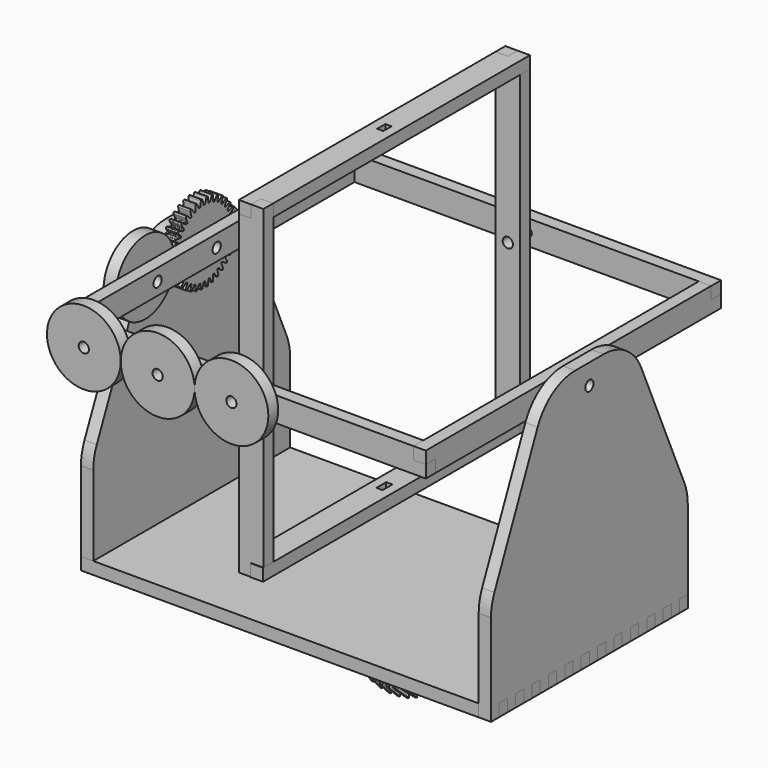
from build123d import *

# Parameters (mm, degrees)
F1_DEPTH  = 6
F2_R      = 2.5
F3_DEPTH  = 6
F4_R      = 2.5
F5_DEPTH  = 6
F6_R      = 2.5
F7_DEPTH  = 6
F8_R      = 2.5
F9_DEPTH  = 6
F10_R     = 2.5
F11_DEPTH = 6
F12_R     = 2.5
F13_DEPTH = 6
F14_R     = 2.5
F15_DEPTH = 6
F16_R     = 2.5
F17_DEPTH = 6
F18_W     = 3
F18_H     = 5
F19_DEPTH = 6
F20_R     = 2.5
F21_DEPTH = 6
F22_W     = 3
F22_H     = 6
F23_DEPTH = 6
F26_R     = 18
F26_R_2   = 2.5
F27_DEPTH = 6
F28_R     = 18
F28_R_2   = 2.5
F29_DEPTH = 6
F30_R     = 18
F30_R_2   = 2.5
F31_DEPTH = 6
F32_R     = 18
F32_R_2   = 2.5
F33_DEPTH = 6
F40_R     = 2.5
F41_DEPTH = 25


# Not quite as in the source:
# - a feature of the source that left no trace in its solid (it failed there, or was rolled back) is left out


with BuildPart() as f1:
    # F0 (on Top) → F1 (new body)
    with BuildSketch(Plane.XY):
        Polygon((100, 55), (100, 60), (-94, 60), (-94, 55), (-100, 55), (-100, 50), (-94, 50), (-94, 45), (-100, 45), (-100, 40), (-94, 40), (-94, 35), (-100, 35), (-100, 30), (-94, 30), (-94, 25), (-100, 25), (-100, 20), (-94, 20), (-94, 15), (-100, 15), (-100, 10), (-94, 10), (-94, 5), (-100, 5), (-100, 0), (-94, 0), (-94, -5), (-100, -5), (-100, -10), (-94, -10), (-94, -15), (-100, -15), (-100, -20), (-94, -20), (-94, -25), (-100, -25), (-100, -30), (-94.03226391, -29.3786096558), (-94.03226391, -34.3786096558), (-100, -35), (-100, -40), (-94, -40), (-94, -45), (-100, -45), (-100, -50), (-94, -50), (-94, -55), (-100, -55), (-100, -60), (94, -60), (94, -55), (100, -55), (100, -50), (94, -50), (94, -45), (100, -45), (100, -40), (94, -40), (94, -35), (100, -35), (100, -30), (94, -30), (94, -25), (100, -25), (100, -20), (94, -20), (94, -15), (100, -15), (100, -10), (94, -10), (94, -5), (100, -5), (100, 0), (94, 0), (94, 5), (100, 5), (100, 10), (94, 10), (94, 15), (100, 15), (100, 20), (94, 20), (94, 25), (100, 25), (100, 30), (94, 30), (94, 35), (100, 35), (100, 40), (94, 40), (94, 45), (100, 45), (100, 50), (94, 50), (94, 55), align=None)
    extrude(amount=F1_DEPTH)


with BuildPart() as f3:
    # F2 (on face) → F3 (new body)
    with BuildSketch(Plane.YZ.offset(100)):
        with BuildLine():
            Line((50, 0), (55, 0))
            Line((55, 0), (55, 6))
            Line((55, 6), (60, 6))
            Line((60, 6), (60, 44.7705385837))
            ThreePointArc((60, 44.7705385837), (59.4703732533, 49.8892134945), (57.9039333726, 54.7910094342))
            Line((57.9039333726, 54.7910094342), (31.5535440029, 115.0204708505))
            ThreePointArc((31.5535440029, 115.0204708505), (22.3333277558, 125.9226166057), (8.6496106304, 130))
            Line((8.6496106304, 130), (-8.6496106304, 130))
            ThreePointArc((-8.6496106304, 130), (-22.3333277558, 125.9226166057), (-31.5535440029, 115.0204708505))
            Line((-31.5535440029, 115.0204708505), (-57.9039333726, 54.7910094342))
            ThreePointArc((-57.9039333726, 54.7910094342), (-59.4703732533, 49.8892134945), (-60, 44.7705385837))
            Line((-60, 44.7705385837), (-60, 0))
            Line((-60, 0), (-55, 0))
            Line((-55, 0), (-55, 6))
            Line((-55, 6), (-50, 6))
            Line((-50, 6), (-50, 0))
            Line((-50, 0), (-45, 0))
            Line((-45, 0), (-45, 6))
            Line((-45, 6), (-40, 6))
            Line((-40, 6), (-40, 0))
            Line((-40, 0), (-35, 0))
            Line((-35, 0), (-35, 6))
            Line((-35, 6), (-30, 6))
            Line((-30, 6), (-30, 0))
            Line((-30, 0), (-25, 0))
            Line((-25, 0), (-25, 6))
            Line((-25, 6), (-20, 6))
            Line((-20, 6), (-20, 0))
            Line((-20, 0), (-15, 0))
            Line((-15, 0), (-15, 6))
            Line((-15, 6), (-10, 6))
            Line((-10, 6), (-10, 0))
            Line((-10, 0), (-5, 0))
            Line((-5, 0), (-5, 6))
            Line((-5, 6), (0, 6))
            Line((0, 6), (0, 0))
            Line((0, 0), (5, 0))
            Line((5, 0), (5, 6))
            Line((5, 6), (10, 6))
            Line((10, 6), (10, 0))
            Line((10, 0), (15, 0))
            Line((15, 0), (15, 6))
            Line((15, 6), (20, 6))
            Line((20, 6), (20, 0))
            Line((20, 0), (25, 0))
            Line((25, 0), (25, 6))
            Line((25, 6), (30, 6))
            Line((30, 6), (30, 0))
            Line((30, 0), (35, 0))
            Line((35, 0), (35, 6))
            Line((35, 6), (40, 6))
            Line((40, 6), (40, 0))
            Line((40, 0), (45, 0))
            Line((45, 0), (45, 6))
            Line((45, 6), (50, 6))
            Line((50, 6), (50, 0))
        make_face()
        with Locations((0, 120)):
            Circle(F2_R, mode=Mode.SUBTRACT)
    extrude(amount=-F3_DEPTH)


with BuildPart() as f5:
    # F4 (on face) → F5 (new body)
    with BuildSketch(Plane(origin=(-100, 0, 0), x_dir=(0, -1, 0), z_dir=(-1, 0, 0))):
        with BuildLine():
            Line((50, 0), (55, 0))
            Line((55, 0), (55, 6))
            Line((55, 6), (60, 6))
            Line((60, 6), (60, 45.0277700469))
            ThreePointArc((60, 45.0277700469), (59.4580269805, 50.2051164927), (57.8556067024, 55.1579843716))
            Line((57.8556067024, 55.1579843716), (31.2743152553, 115.1302143247))
            ThreePointArc((31.2743152553, 115.1302143247), (22.0522085049, 125.9553735128), (8.4187085529, 130))
            Line((8.4187085529, 130), (-8.9065918714, 130))
            ThreePointArc((-8.9065918714, 130), (-22.6250646146, 125.8998446308), (-31.8437077839, 114.9442804474))
            Line((-31.8437077839, 114.9442804474), (-57.9371159125, 54.7581734726))
            ThreePointArc((-57.9371159125, 54.7581734726), (-59.4788469685, 49.8918897851), (-60, 44.8138930252))
            Line((-60, 44.8138930252), (-60, 0))
            Line((-60, 0), (-55, 0))
            Line((-55, 0), (-55, 6))
            Line((-55, 6), (-50, 6))
            Line((-50, 6), (-50, 0))
            Line((-50, 0), (-45, 0))
            Line((-45, 0), (-45, 6))
            Line((-45, 6), (-40, 6))
            Line((-40, 6), (-40, 0))
            Line((-40, 0), (-35, 0))
            Line((-35, 0), (-35, 6))
            Line((-35, 6), (-30, 6))
            Line((-30, 6), (-30, 0))
            Line((-30, 0), (-25, 0))
            Line((-25, 0), (-25, 6))
            Line((-25, 6), (-20, 6))
            Line((-20, 6), (-20, 0))
            Line((-20, 0), (-15, 0))
            Line((-15, 0), (-15, 6))
            Line((-15, 6), (-10, 6))
            Line((-10, 6), (-10, 0))
            Line((-10, 0), (-5, 0))
            Line((-5, 0), (-5, 6))
            Line((-5, 6), (0, 6))
            Line((0, 6), (0, 0))
            Line((0, 0), (5, 0))
            Line((5, 0), (5, 6))
            Line((5, 6), (10, 6))
            Line((10, 6), (10, 0))
            Line((10, 0), (15, 0))
            Line((15, 0), (15, 6))
            Line((15, 6), (20, 6))
            Line((20, 6), (20, 0))
            Line((20, 0), (25, 0))
            Line((25, 0), (25, 6))
            Line((25, 6), (30, 6))
            Line((30, 6), (30, 0))
            Line((30, 0), (35, 0))
            Line((35, 0), (35, 6))
            Line((35, 6), (40, 6))
            Line((40, 6), (40, 0))
            Line((40, 0), (45, 0))
            Line((45, 0), (45, 6))
            Line((45, 6), (50, 6))
            Line((50, 6), (50, 0))
        make_face()
        with Locations((-0.2439416593, 120)):
            Circle(F4_R, mode=Mode.SUBTRACT)
    extrude(amount=-F5_DEPTH)


with BuildPart() as f7:
    # F6 (on face) → F7 (new body)
    with BuildSketch(Plane.YZ.offset(-94)):
        with BuildLine():
            ThreePointArc((-0.9074454432, 138.9766193212), (-1.1059043827, 139.2442584986), (-1.4284580066, 139.3277799904))
            ThreePointArc((-1.4284580066, 139.3277799904), (-1.44687975, 139.326177143), (-1.4652999573, 139.3245567374))
            ThreePointArc((-1.4652999573, 139.3245567374), (-1.7684499121, 139.1862932757), (-1.9174187589, 138.8882581056))
            Line((-1.9174187589, 138.8882581056), (-2.2042135214, 136.5840744477))
            ThreePointArc((-2.2042135214, 136.5840744477), (-2.3348708966, 136.3046577179), (-2.6046356928, 136.1550849487))
            ThreePointArc((-2.6046356928, 136.1550849487), (-2.9092885812, 136.2033723819), (-3.1276325025, 136.4212507668))
            Line((-3.1276325025, 136.4212507668), (-4.1852086494, 138.4883855613))
            ThreePointArc((-4.1852086494, 138.4883855613), (-4.427127607, 138.7174966651), (-4.7592842715, 138.7437384288))
            ThreePointArc((-4.7592842715, 138.7437384288), (-4.7771478157, 138.73896103), (-4.7950067982, 138.7341666066))
            ThreePointArc((-4.7950067982, 138.7341666066), (-5.0695420259, 138.5453622404), (-5.164494437, 138.2259867254))
            Line((-5.164494437, 138.2259867254), (-5.0468148493, 135.9070074068))
            ThreePointArc((-5.0468148493, 135.9070074068), (-5.1269670395, 135.6091472299), (-5.3666604635, 135.415002642))
            ThreePointArc((-5.3666604635, 135.415002642), (-5.6750700147, 135.4096540616), (-5.9279309858, 135.5863073602))
            Line((-5.9279309858, 135.5863073602), (-7.3283943647, 137.4383915618))
            ThreePointArc((-7.3283943647, 137.4383915618), (-7.6064227554, 137.6220131669), (-7.9380900483, 137.5901778597))
            ThreePointArc((-7.9380900483, 137.5901778597), (-7.9548526185, 137.5823710685), (-7.97160774, 137.5745483034))
            ThreePointArc((-7.97160774, 137.5745483034), (-8.2091866266, 137.3409397577), (-8.247237521, 137.0099279613))
            Line((-8.247237521, 137.0099279613), (-7.728659218, 134.7466139953))
            ThreePointArc((-7.728659218, 134.7466139953), (-7.7558708394, 134.439360702), (-7.9582099279, 134.2065432803))
            ThreePointArc((-7.9582099279, 134.2065432803), (-8.2610052737, 134.1477212004), (-8.5407002418, 134.2777818916))
            Line((-8.5407002418, 134.2777818916), (-10.2414984817, 135.8585408589))
            ThreePointArc((-10.2414984817, 135.8585408589), (-10.5471885535, 135.9910937158), (-10.8682889319, 135.9021486375))
            ThreePointArc((-10.8682889319, 135.9021486375), (-10.883441206, 135.8915496592), (-10.8985833706, 135.8809362432))
            ThreePointArc((-10.8985833706, 135.8809362432), (-11.0919872018, 135.6096215955), (-11.0719804224, 135.2770311436))
            Line((-11.0719804224, 135.2770311436), (-10.1682601434, 133.1381521796))
            ThreePointArc((-10.1682601434, 133.1381521796), (-10.1417043847, 132.8308415058), (-10.3005411667, 132.5664252899))
            ThreePointArc((-10.3005411667, 132.5664252899), (-10.5885220239, 132.4559169895), (-10.886552599, 132.5354332451))
            Line((-10.886552599, 132.5354332451), (-12.8360078059, 133.7968364168))
            ThreePointArc((-12.8360078059, 133.7968364168), (-13.1600713207, 133.8742929741), (-13.4608483121, 133.7309406758))
            ThreePointArc((-13.4608483121, 133.7309406758), (-13.4739298958, 133.717871555), (-13.4869990165, 133.7047899713))
            ThreePointArc((-13.4869990165, 133.7047899713), (-13.6303513148, 133.40401298), (-13.5528947575, 133.0799494651))
            Line((-13.5528947575, 133.0799494651), (-12.2914915858, 131.1304942582))
            ThreePointArc((-12.2914915858, 131.1304942582), (-12.2119753303, 130.8324636832), (-12.3224836306, 130.5444828259))
            ThreePointArc((-12.3224836306, 130.5444828259), (-12.5868998465, 130.3856460439), (-12.8942105204, 130.4122018027))
            Line((-12.8942105204, 130.4122018027), (-15.0330894843, 131.3159220817))
            ThreePointArc((-15.0330894843, 131.3159220817), (-15.3656799363, 131.335928861), (-15.6369945839, 131.1425250298))
            ThreePointArc((-15.6369945839, 131.1425250298), (-15.647608, 131.1273828652), (-15.6582069782, 131.1122305911))
            ThreePointArc((-15.6582069782, 131.1122305911), (-15.7471520566, 130.7911302128), (-15.6145991996, 130.4854401409))
            Line((-15.6145991996, 130.4854401409), (-14.0338402323, 128.7846419011))
            ThreePointArc((-14.0338402323, 128.7846419011), (-13.9037795411, 128.504946933), (-13.962601621, 128.2021515871))
            ThreePointArc((-13.962601621, 128.2021515871), (-14.1954190427, 127.9998124987), (-14.502672336, 127.9726008773))
            Line((-14.502672336, 127.9726008773), (-16.7659863021, 128.4911791803))
            ThreePointArc((-16.7659863021, 128.4911791803), (-17.0969980985, 128.4531282858), (-17.3306066441, 128.2155493993))
            ThreePointArc((-17.3306066441, 128.2155493993), (-17.3384294093, 128.1987942778), (-17.3462362005, 128.1820317075))
            ThreePointArc((-17.3462362005, 128.1820317075), (-17.3780715077, 127.8503644147), (-17.1944499025, 127.5723360239))
            Line((-17.1944499025, 127.5723360239), (-15.342365701, 126.171872645))
            ThreePointArc((-15.342365701, 126.171872645), (-15.1657124024, 125.919011674), (-15.1710609827, 125.6106021228))
            ThreePointArc((-15.1710609827, 125.6106021228), (-15.3652055707, 125.3709086988), (-15.6630657476, 125.2907565086))
            Line((-15.6630657476, 125.2907565086), (-17.9820450661, 125.4084360962))
            ThreePointArc((-17.9820450661, 125.4084360962), (-18.3014205811, 125.3134836851), (-18.4902249473, 125.0389484574))
            ThreePointArc((-18.4902249473, 125.0389484574), (-18.4950193708, 125.021089475), (-18.4997967695, 125.0032259308))
            ThreePointArc((-18.4997967695, 125.0032259308), (-18.4735550058, 124.6710692663), (-18.2444439021, 124.4291503086))
            Line((-18.2444439021, 124.4291503086), (-16.1773091075, 123.3715741617))
            ThreePointArc((-16.1773091075, 123.3715741617), (-15.9594307227, 123.1532302404), (-15.9111432895, 122.8485773521))
            ThreePointArc((-15.9111432895, 122.8485773521), (-16.0607160587, 122.5788125559), (-16.3401327884, 122.4481551806))
            Line((-16.3401327884, 122.4481551806), (-18.6443164463, 122.1613604182))
            ThreePointArc((-18.6443164463, 122.1613604182), (-18.9423516165, 122.0123915714), (-19.0806150781, 121.7092416166))
            ThreePointArc((-19.0806150781, 121.7092416166), (-19.0822354837, 121.6908214093), (-19.0838383312, 121.6723996659))
            ThreePointArc((-19.0838383312, 121.6723996659), (-19.0003168394, 121.3498460419), (-18.7326776619, 121.1513871025))
            Line((-18.7326776619, 121.1513871025), (-16.5133011191, 120.4688321037))
            ThreePointArc((-16.5133011191, 120.4688321037), (-16.2608177724, 120.2916395016), (-16.160361515, 120))
            ThreePointArc((-16.160361515, 120), (-16.2608177724, 119.7083604984), (-16.5133011191, 119.5311678963))
            Line((-16.5133011191, 119.5311678963), (-18.7326776619, 118.8486128975))
            ThreePointArc((-18.7326776619, 118.8486128975), (-19.0003168394, 118.6501539581), (-19.0838383312, 118.3276003341))
            ThreePointArc((-19.0838383312, 118.3276003341), (-19.0822354837, 118.3091785907), (-19.0806150781, 118.2907583834))
            ThreePointArc((-19.0806150781, 118.2907583834), (-18.9423516165, 117.9876084286), (-18.6443164463, 117.8386395818))
            Line((-18.6443164463, 117.8386395818), (-16.3401327884, 117.5518448194))
            ThreePointArc((-16.3401327884, 117.5518448194), (-16.0607160587, 117.4211874442), (-15.9111432895, 117.1514226479))
            ThreePointArc((-15.9111432895, 117.1514226479), (-15.9594307227, 116.8467697596), (-16.1773091075, 116.6284258383))
            Line((-16.1773091075, 116.6284258383), (-18.2444439021, 115.5708496914))
            ThreePointArc((-18.2444439021, 115.5708496914), (-18.4735550058, 115.3289307337), (-18.4997967695, 114.9967740692))
            ThreePointArc((-18.4997967695, 114.9967740692), (-18.4950193708, 114.978910525), (-18.4902249473, 114.9610515426))
            ThreePointArc((-18.4902249473, 114.9610515426), (-18.3014205811, 114.6865163149), (-17.9820450661, 114.5915639038))
            Line((-17.9820450661, 114.5915639038), (-15.6630657476, 114.7092434914))
            ThreePointArc((-15.6630657476, 114.7092434914), (-15.3652055707, 114.6290913012), (-15.1710609827, 114.3893978772))
            ThreePointArc((-15.1710609827, 114.3893978772), (-15.1657124024, 114.080988326), (-15.342365701, 113.828127355))
            Line((-15.342365701, 113.828127355), (-17.1944499025, 112.4276639761))
            ThreePointArc((-17.1944499025, 112.4276639761), (-17.3780715077, 112.1496355853), (-17.3462362005, 111.8179682925))
            ThreePointArc((-17.3462362005, 111.8179682925), (-17.3384294093, 111.8012057222), (-17.3306066441, 111.7844506007))
            ThreePointArc((-17.3306066441, 111.7844506007), (-17.0969980985, 111.5468717142), (-16.7659863021, 111.5088208197))
            Line((-16.7659863021, 111.5088208197), (-14.502672336, 112.0273991227))
            ThreePointArc((-14.502672336, 112.0273991227), (-14.1954190427, 112.0001875013), (-13.962601621, 111.7978484129))
            ThreePointArc((-13.962601621, 111.7978484129), (-13.9037795411, 111.495053067), (-14.0338402323, 111.2153580989))
            Line((-14.0338402323, 111.2153580989), (-15.6145991996, 109.5145598591))
            ThreePointArc((-15.6145991996, 109.5145598591), (-15.7471520566, 109.2088697872), (-15.6582069782, 108.8877694089))
            ThreePointArc((-15.6582069782, 108.8877694089), (-15.647608, 108.8726171348), (-15.6369945839, 108.8574749702))
            ThreePointArc((-15.6369945839, 108.8574749702), (-15.3656799363, 108.664071139), (-15.0330894843, 108.6840779183))
            Line((-15.0330894843, 108.6840779183), (-12.8942105204, 109.5877981973))
            ThreePointArc((-12.8942105204, 109.5877981973), (-12.5868998465, 109.6143539561), (-12.3224836306, 109.4555171741))
            ThreePointArc((-12.3224836306, 109.4555171741), (-12.2119753303, 109.1675363168), (-12.2914915858, 108.8695057418))
            Line((-12.2914915858, 108.8695057418), (-13.5528947575, 106.9200505349))
            ThreePointArc((-13.5528947575, 106.9200505349), (-13.6303513148, 106.59598702), (-13.4869990165, 106.2952100287))
            ThreePointArc((-13.4869990165, 106.2952100287), (-13.4739298958, 106.282128445), (-13.4608483121, 106.2690593242))
            ThreePointArc((-13.4608483121, 106.2690593242), (-13.1600713207, 106.1257070259), (-12.8360078059, 106.2031635832))
            Line((-12.8360078059, 106.2031635832), (-10.886552599, 107.4645667549))
            ThreePointArc((-10.886552599, 107.4645667549), (-10.5885220239, 107.5440830105), (-10.3005411667, 107.4335747102))
            ThreePointArc((-10.3005411667, 107.4335747102), (-10.1417043847, 107.1691584942), (-10.1682601434, 106.8618478204))
            Line((-10.1682601434, 106.8618478204), (-11.0719804224, 104.7229688564))
            ThreePointArc((-11.0719804224, 104.7229688564), (-11.0919872018, 104.3903784045), (-10.8985833706, 104.1190637568))
            ThreePointArc((-10.8985833706, 104.1190637568), (-10.883441206, 104.1084503408), (-10.8682889319, 104.0978513625))
            ThreePointArc((-10.8682889319, 104.0978513625), (-10.5471885535, 104.0089062842), (-10.2414984817, 104.1414591411))
            Line((-10.2414984817, 104.1414591411), (-8.5407002418, 105.7222181084))
            ThreePointArc((-8.5407002418, 105.7222181084), (-8.2610052737, 105.8522787996), (-7.9582099279, 105.7934567197))
            ThreePointArc((-7.9582099279, 105.7934567197), (-7.7558708394, 105.560639298), (-7.728659218, 105.2533860047))
            Line((-7.728659218, 105.2533860047), (-8.247237521, 102.9900720387))
            ThreePointArc((-8.247237521, 102.9900720387), (-8.2091866266, 102.6590602423), (-7.97160774, 102.4254516966))
            ThreePointArc((-7.97160774, 102.4254516966), (-7.9548526185, 102.4176289315), (-7.9380900483, 102.4098221403))
            ThreePointArc((-7.9380900483, 102.4098221403), (-7.6064227554, 102.3779868331), (-7.3283943647, 102.5616084382))
            Line((-7.3283943647, 102.5616084382), (-5.9279309858, 104.4136926398))
            ThreePointArc((-5.9279309858, 104.4136926398), (-5.6750700147, 104.5903459384), (-5.3666604636, 104.5849973581))
            ThreePointArc((-5.3666604636, 104.5849973581), (-5.1269670395, 104.3908527701), (-5.0468148493, 104.0929925932))
            Line((-5.0468148493, 104.0929925932), (-5.164494437, 101.7740132746))
            ThreePointArc((-5.164494437, 101.7740132746), (-5.0695420259, 101.4546377596), (-4.7950067982, 101.2658333934))
            ThreePointArc((-4.7950067982, 101.2658333934), (-4.7771478157, 101.26103897), (-4.7592842715, 101.2562615712))
            ThreePointArc((-4.7592842715, 101.2562615712), (-4.427127607, 101.2825033349), (-4.1852086494, 101.5116144387))
            Line((-4.1852086494, 101.5116144387), (-3.1276325025, 103.5787492332))
            ThreePointArc((-3.1276325025, 103.5787492332), (-2.9092885812, 103.7966276181), (-2.6046356928, 103.8449150513))
            ThreePointArc((-2.6046356928, 103.8449150513), (-2.3348708966, 103.6953422821), (-2.2042135214, 103.4159255523))
            Line((-2.2042135214, 103.4159255523), (-1.9174187589, 101.1117418944))
            ThreePointArc((-1.9174187589, 101.1117418944), (-1.7684499121, 100.8137067243), (-1.4652999573, 100.6754432626))
            ThreePointArc((-1.4652999573, 100.6754432626), (-1.44687975, 100.673822857), (-1.4284580066, 100.6722200096))
            ThreePointArc((-1.4284580066, 100.6722200096), (-1.1059043827, 100.7557415014), (-0.9074454432, 101.0233806788))
            Line((-0.9074454432, 101.0233806788), (-0.2248904444, 103.2427572216))
            ThreePointArc((-0.2248904444, 103.2427572216), (-0.0476978424, 103.4952405683), (0.2439416592, 103.5956968258))
            ThreePointArc((0.2439416592, 103.5956968258), (0.5355811609, 103.4952405683), (0.7127737629, 103.2427572216))
            Line((0.7127737629, 103.2427572216), (1.3953287617, 101.0233806788))
            ThreePointArc((1.3953287617, 101.0233806788), (1.5937877012, 100.7557415014), (1.9163413251, 100.6722200096))
            ThreePointArc((1.9163413251, 100.6722200096), (1.9347630686, 100.673822857), (1.9531832758, 100.6754432626))
            ThreePointArc((1.9531832758, 100.6754432626), (2.2563332306, 100.8137067243), (2.4053020774, 101.1117418944))
            Line((2.4053020774, 101.1117418944), (2.6920968399, 103.4159255523))
            ThreePointArc((2.6920968399, 103.4159255523), (2.8227542151, 103.6953422821), (3.0925190113, 103.8449150513))
            ThreePointArc((3.0925190113, 103.8449150513), (3.3971718997, 103.7966276181), (3.615515821, 103.5787492332))
            Line((3.615515821, 103.5787492332), (4.6730919679, 101.5116144387))
            ThreePointArc((4.6730919679, 101.5116144387), (4.9150109255, 101.2825033349), (5.24716759, 101.2562615712))
            ThreePointArc((5.24716759, 101.2562615712), (5.2650311342, 101.26103897), (5.2828901167, 101.2658333934))
            ThreePointArc((5.2828901167, 101.2658333934), (5.5574253444, 101.4546377596), (5.6523777555, 101.7740132746))
            Line((5.6523777555, 101.7740132746), (5.5346981678, 104.0929925932))
            ThreePointArc((5.5346981678, 104.0929925932), (5.614850358, 104.3908527701), (5.8545437821, 104.584997358))
            ThreePointArc((5.8545437821, 104.584997358), (6.1629533332, 104.5903459384), (6.4158143043, 104.4136926398))
            Line((6.4158143043, 104.4136926398), (7.8162776832, 102.5616084382))
            ThreePointArc((7.8162776832, 102.5616084382), (8.0943060739, 102.3779868331), (8.4259733668, 102.4098221403))
            ThreePointArc((8.4259733668, 102.4098221403), (8.442735937, 102.4176289315), (8.4594910585, 102.4254516966))
            ThreePointArc((8.4594910585, 102.4254516966), (8.6970699451, 102.6590602423), (8.7351208395, 102.9900720387))
            Line((8.7351208395, 102.9900720387), (8.2165425365, 105.2533860047))
            ThreePointArc((8.2165425365, 105.2533860047), (8.2437541579, 105.560639298), (8.4460932464, 105.7934567197))
            ThreePointArc((8.4460932464, 105.7934567197), (8.7488885922, 105.8522787996), (9.0285835603, 105.7222181084))
            Line((9.0285835603, 105.7222181084), (10.7293818002, 104.1414591411))
            ThreePointArc((10.7293818002, 104.1414591411), (11.0350718721, 104.0089062842), (11.3561722504, 104.0978513625))
            ThreePointArc((11.3561722504, 104.0978513625), (11.3713245245, 104.1084503408), (11.3864666891, 104.1190637568))
            ThreePointArc((11.3864666891, 104.1190637568), (11.5798705203, 104.3903784045), (11.5598637409, 104.7229688564))
            Line((11.5598637409, 104.7229688564), (10.6561434619, 106.8618478204))
            ThreePointArc((10.6561434619, 106.8618478204), (10.6295877032, 107.1691584942), (10.7884244852, 107.4335747101))
            ThreePointArc((10.7884244852, 107.4335747101), (11.0764053424, 107.5440830105), (11.3744359175, 107.4645667549))
            Line((11.3744359175, 107.4645667549), (13.3238911244, 106.2031635832))
            ThreePointArc((13.3238911244, 106.2031635832), (13.6479546392, 106.1257070259), (13.9487316306, 106.2690593242))
            ThreePointArc((13.9487316306, 106.2690593242), (13.9618132143, 106.282128445), (13.9748823351, 106.2952100287))
            ThreePointArc((13.9748823351, 106.2952100287), (14.1182346333, 106.59598702), (14.040778076, 106.9200505349))
            Line((14.040778076, 106.9200505349), (12.7793749043, 108.8695057418))
            ThreePointArc((12.7793749043, 108.8695057418), (12.6998586488, 109.1675363168), (12.8103669491, 109.4555171741))
            ThreePointArc((12.8103669491, 109.4555171741), (13.074783165, 109.6143539561), (13.3820938389, 109.5877981973))
            Line((13.3820938389, 109.5877981973), (15.5209728028, 108.6840779183))
            ThreePointArc((15.5209728028, 108.6840779183), (15.8535632548, 108.664071139), (16.1248779024, 108.8574749702))
            ThreePointArc((16.1248779024, 108.8574749702), (16.1354913185, 108.8726171348), (16.1460902968, 108.8877694089))
            ThreePointArc((16.1460902968, 108.8877694089), (16.2350353751, 109.2088697872), (16.1024825181, 109.5145598591))
            Line((16.1024825181, 109.5145598591), (14.5217235509, 111.2153580989))
            ThreePointArc((14.5217235509, 111.2153580989), (14.3916628596, 111.495053067), (14.4504849395, 111.7978484129))
            ThreePointArc((14.4504849395, 111.7978484129), (14.6833023613, 112.0001875013), (14.9905556545, 112.0273991227))
            Line((14.9905556545, 112.0273991227), (17.2538696206, 111.5088208197))
            ThreePointArc((17.2538696206, 111.5088208197), (17.584881417, 111.5468717142), (17.8184899626, 111.7844506007))
            ThreePointArc((17.8184899626, 111.7844506007), (17.8263127278, 111.8012057222), (17.834119519, 111.8179682925))
            ThreePointArc((17.834119519, 111.8179682925), (17.8659548262, 112.1496355853), (17.682333221, 112.4276639761))
            Line((17.682333221, 112.4276639761), (15.8302490195, 113.828127355))
            ThreePointArc((15.8302490195, 113.828127355), (15.6535957209, 114.080988326), (15.6589443012, 114.3893978772))
            ThreePointArc((15.6589443012, 114.3893978772), (15.8530888892, 114.6290913012), (16.1509490661, 114.7092434914))
            Line((16.1509490661, 114.7092434914), (18.4699283846, 114.5915639038))
            ThreePointArc((18.4699283846, 114.5915639038), (18.7893038996, 114.6865163149), (18.9781082658, 114.9610515426))
            ThreePointArc((18.9781082658, 114.9610515426), (18.9829026893, 114.978910525), (18.987680088, 114.9967740692))
            ThreePointArc((18.987680088, 114.9967740692), (18.9614383244, 115.3289307337), (18.7323272206, 115.5708496914))
            Line((18.7323272206, 115.5708496914), (16.6651924261, 116.6284258383))
            ThreePointArc((16.6651924261, 116.6284258383), (16.4473140412, 116.8467697596), (16.399026608, 117.1514226479))
            ThreePointArc((16.399026608, 117.1514226479), (16.5485993772, 117.4211874441), (16.8280161069, 117.5518448194))
            Line((16.8280161069, 117.5518448194), (19.1321997648, 117.8386395818))
            ThreePointArc((19.1321997648, 117.8386395818), (19.430234935, 117.9876084286), (19.5684983966, 118.2907583834))
            ThreePointArc((19.5684983966, 118.2907583834), (19.5701188022, 118.3091785907), (19.5717216497, 118.3276003341))
            ThreePointArc((19.5717216497, 118.3276003341), (19.4882001579, 118.6501539581), (19.2205609804, 118.8486128975))
            Line((19.2205609804, 118.8486128975), (17.0011844376, 119.5311678963))
            ThreePointArc((17.0011844376, 119.5311678963), (16.7487010909, 119.7083604984), (16.6482448335, 120))
            ThreePointArc((16.6482448335, 120), (16.7487010909, 120.2916395016), (17.0011844376, 120.4688321037))
            Line((17.0011844376, 120.4688321037), (19.2205609804, 121.1513871025))
            ThreePointArc((19.2205609804, 121.1513871025), (19.4882001579, 121.3498460419), (19.5717216497, 121.6723996659))
            ThreePointArc((19.5717216497, 121.6723996659), (19.5701188022, 121.6908214093), (19.5684983966, 121.7092416166))
            ThreePointArc((19.5684983966, 121.7092416166), (19.430234935, 122.0123915714), (19.1321997648, 122.1613604182))
            Line((19.1321997648, 122.1613604182), (16.8280161069, 122.4481551806))
            ThreePointArc((16.8280161069, 122.4481551806), (16.5485993772, 122.5788125558), (16.399026608, 122.8485773521))
            ThreePointArc((16.399026608, 122.8485773521), (16.4473140412, 123.1532302404), (16.6651924261, 123.3715741617))
            Line((16.6651924261, 123.3715741617), (18.7323272206, 124.4291503086))
            ThreePointArc((18.7323272206, 124.4291503086), (18.9614383244, 124.6710692663), (18.987680088, 125.0032259308))
            ThreePointArc((18.987680088, 125.0032259308), (18.9829026893, 125.021089475), (18.9781082658, 125.0389484574))
            ThreePointArc((18.9781082658, 125.0389484574), (18.7893038996, 125.3134836851), (18.4699283846, 125.4084360962))
            Line((18.4699283846, 125.4084360962), (16.1509490661, 125.2907565086))
            ThreePointArc((16.1509490661, 125.2907565086), (15.8530888892, 125.3709086988), (15.6589443012, 125.6106021228))
            ThreePointArc((15.6589443012, 125.6106021228), (15.6535957209, 125.919011674), (15.8302490195, 126.171872645))
            Line((15.8302490195, 126.171872645), (17.682333221, 127.5723360239))
            ThreePointArc((17.682333221, 127.5723360239), (17.8659548262, 127.8503644147), (17.834119519, 128.1820317075))
            ThreePointArc((17.834119519, 128.1820317075), (17.8263127278, 128.1987942778), (17.8184899626, 128.2155493993))
            ThreePointArc((17.8184899626, 128.2155493993), (17.584881417, 128.4531282858), (17.2538696206, 128.4911791803))
            Line((17.2538696206, 128.4911791803), (14.9905556545, 127.9726008773))
            ThreePointArc((14.9905556545, 127.9726008773), (14.6833023613, 127.9998124987), (14.4504849395, 128.2021515871))
            ThreePointArc((14.4504849395, 128.2021515871), (14.3916628596, 128.504946933), (14.5217235509, 128.7846419011))
            Line((14.5217235509, 128.7846419011), (16.1024825181, 130.4854401409))
            ThreePointArc((16.1024825181, 130.4854401409), (16.2350353751, 130.7911302128), (16.1460902968, 131.1122305911))
            ThreePointArc((16.1460902968, 131.1122305911), (16.1354913185, 131.1273828652), (16.1248779024, 131.1425250298))
            ThreePointArc((16.1248779024, 131.1425250298), (15.8535632548, 131.335928861), (15.5209728028, 131.3159220817))
            Line((15.5209728028, 131.3159220817), (13.3820938389, 130.4122018027))
            ThreePointArc((13.3820938389, 130.4122018027), (13.0747831651, 130.3856460439), (12.8103669491, 130.5444828259))
            ThreePointArc((12.8103669491, 130.5444828259), (12.6998586488, 130.8324636832), (12.7793749043, 131.1304942582))
            Line((12.7793749043, 131.1304942582), (14.040778076, 133.0799494651))
            ThreePointArc((14.040778076, 133.0799494651), (14.1182346333, 133.40401298), (13.9748823351, 133.7047899713))
            ThreePointArc((13.9748823351, 133.7047899713), (13.9618132143, 133.717871555), (13.9487316306, 133.7309406758))
            ThreePointArc((13.9487316306, 133.7309406758), (13.6479546392, 133.8742929741), (13.3238911244, 133.7968364168))
            Line((13.3238911244, 133.7968364168), (11.3744359175, 132.5354332451))
            ThreePointArc((11.3744359175, 132.5354332451), (11.0764053424, 132.4559169895), (10.7884244852, 132.5664252898))
            ThreePointArc((10.7884244852, 132.5664252898), (10.6295877032, 132.8308415058), (10.6561434619, 133.1381521796))
            Line((10.6561434619, 133.1381521796), (11.5598637409, 135.2770311436))
            ThreePointArc((11.5598637409, 135.2770311436), (11.5798705203, 135.6096215955), (11.3864666891, 135.8809362432))
            ThreePointArc((11.3864666891, 135.8809362432), (11.3713245245, 135.8915496592), (11.3561722504, 135.9021486375))
            ThreePointArc((11.3561722504, 135.9021486375), (11.0350718721, 135.9910937158), (10.7293818002, 135.8585408589))
            Line((10.7293818002, 135.8585408589), (9.0285835603, 134.2777818916))
            ThreePointArc((9.0285835603, 134.2777818916), (8.7488885923, 134.1477212004), (8.4460932464, 134.2065432803))
            ThreePointArc((8.4460932464, 134.2065432803), (8.2437541579, 134.439360702), (8.2165425365, 134.7466139953))
            Line((8.2165425365, 134.7466139953), (8.7351208395, 137.0099279613))
            ThreePointArc((8.7351208395, 137.0099279613), (8.6970699451, 137.3409397577), (8.4594910585, 137.5745483034))
            ThreePointArc((8.4594910585, 137.5745483034), (8.442735937, 137.5823710685), (8.4259733668, 137.5901778597))
            ThreePointArc((8.4259733668, 137.5901778597), (8.0943060739, 137.6220131669), (7.8162776832, 137.4383915618))
            Line((7.8162776832, 137.4383915618), (6.4158143043, 135.5863073602))
            ThreePointArc((6.4158143043, 135.5863073602), (6.1629533332, 135.4096540616), (5.8545437821, 135.4150026419))
            ThreePointArc((5.8545437821, 135.4150026419), (5.614850358, 135.6091472299), (5.5346981678, 135.9070074068))
            Line((5.5346981678, 135.9070074068), (5.6523777555, 138.2259867254))
            ThreePointArc((5.6523777555, 138.2259867254), (5.5574253444, 138.5453622404), (5.2828901167, 138.7341666066))
            ThreePointArc((5.2828901167, 138.7341666066), (5.2650311342, 138.73896103), (5.24716759, 138.7437384288))
            ThreePointArc((5.24716759, 138.7437384288), (4.9150109255, 138.7174966651), (4.6730919679, 138.4883855613))
            Line((4.6730919679, 138.4883855613), (3.615515821, 136.4212507668))
            ThreePointArc((3.615515821, 136.4212507668), (3.3971718997, 136.2033723819), (3.0925190114, 136.1550849487))
            ThreePointArc((3.0925190114, 136.1550849487), (2.8227542151, 136.3046577179), (2.6920968399, 136.5840744477))
            Line((2.6920968399, 136.5840744477), (2.4053020774, 138.8882581056))
            ThreePointArc((2.4053020774, 138.8882581056), (2.2563332306, 139.1862932757), (1.9531832758, 139.3245567374))
            ThreePointArc((1.9531832758, 139.3245567374), (1.9347630686, 139.326177143), (1.9163413251, 139.3277799904))
            ThreePointArc((1.9163413251, 139.3277799904), (1.5937877012, 139.2442584986), (1.3953287617, 138.9766193212))
            Line((1.3953287617, 138.9766193212), (0.7127737629, 136.7572427784))
            ThreePointArc((0.7127737629, 136.7572427784), (0.5355811609, 136.5047594317), (0.2439416593, 136.4043031742))
            ThreePointArc((0.2439416593, 136.4043031742), (-0.0476978424, 136.5047594317), (-0.2248904444, 136.7572427784))
            Line((-0.2248904444, 136.7572427784), (-0.9074454432, 138.9766193212))
        make_face()
        with BuildLine():
            ThreePointArc((-10.2852554216, 107.4207006941), (-10.2928339664, 107.4272140806), (-10.3005411667, 107.4335747102))
            ThreePointArc((-10.3005411667, 107.4335747102), (-10.3081435053, 107.440060309), (-10.3158739393, 107.446392681))
            Line((-10.3158739393, 107.446392681), (-10.3002843799, 107.4338807368))
            Line((-10.3002843799, 107.4338807368), (-10.2852554216, 107.4207006941))
        make_face(mode=Mode.SUBTRACT)
        with BuildLine():
            ThreePointArc((-12.3096656598, 109.4401844015), (-12.3159980317, 109.4479148355), (-12.3224836306, 109.4555171741))
            ThreePointArc((-12.3224836306, 109.4555171741), (-12.3288442602, 109.4632243744), (-12.3353576467, 109.4708029192))
            Line((-12.3353576467, 109.4708029192), (-12.322177604, 109.4557739609))
            Line((-12.322177604, 109.4557739609), (-12.3096656598, 109.4401844015))
        make_face(mode=Mode.SUBTRACT)
        with BuildLine():
            ThreePointArc((-5.3478933889, 104.5781277729), (-5.3572426009, 104.5816563391), (-5.3666604636, 104.5849973581))
            ThreePointArc((-5.3666604636, 104.5849973581), (-5.3760225305, 104.5884916745), (-5.3854525611, 104.5917981936))
            Line((-5.3854525611, 104.5917981936), (-5.3665238301, 104.5853727553))
            Line((-5.3665238301, 104.5853727553), (-5.3478933889, 104.5781277729))
        make_face(mode=Mode.SUBTRACT)
        with BuildLine():
            ThreePointArc((-2.5849608413, 103.8414086988), (-2.5947807468, 103.8432601846), (-2.6046356928, 103.8449150513))
            ThreePointArc((-2.6046356928, 103.8449150513), (-2.6144623106, 103.8467305753), (-2.6243232489, 103.8483493533))
            Line((-2.6243232489, 103.8483493533), (-2.6045663222, 103.8453084715))
            Line((-2.6045663222, 103.8453084715), (-2.5849608413, 103.8414086988))
        make_face(mode=Mode.SUBTRACT)
        with BuildLine():
            ThreePointArc((-7.9409208582, 105.7834326307), (-7.9495153055, 105.7885310637), (-7.9582099279, 105.7934567197))
            ThreePointArc((-7.9582099279, 105.7934567197), (-7.9668229823, 105.7985236555), (-7.9755355785, 105.8034174488))
            Line((-7.9755355785, 105.8034174488), (-7.9580101832, 105.7938026877))
            Line((-7.9580101832, 105.7938026877), (-7.9409208582, 105.7834326307))
        make_face(mode=Mode.SUBTRACT)
        with BuildLine():
            ThreePointArc((-15.1642601472, 114.3706057797), (-15.1675666662, 114.3800358103), (-15.1710609827, 114.3893978772))
            ThreePointArc((-15.1710609827, 114.3893978772), (-15.1744020016, 114.3988157399), (-15.1779305679, 114.4081649519))
            Line((-15.1779305679, 114.4081649519), (-15.1706855855, 114.3895345106))
            Line((-15.1706855855, 114.3895345106), (-15.1642601472, 114.3706057797))
        make_face(mode=Mode.SUBTRACT)
        with BuildLine():
            ThreePointArc((-13.952640892, 111.7805227623), (-13.9575346852, 111.7892353585), (-13.962601621, 111.7978484129))
            ThreePointArc((-13.962601621, 111.7978484129), (-13.967527277, 111.8065430352), (-13.9726257101, 111.8151374826))
            Line((-13.9726257101, 111.8151374826), (-13.9622556531, 111.7980481576))
            Line((-13.9622556531, 111.7980481576), (-13.952640892, 111.7805227623))
        make_face(mode=Mode.SUBTRACT)
        with BuildLine():
            ThreePointArc((-15.9077089874, 117.1317350919), (-15.9093277654, 117.1415960301), (-15.9111432895, 117.1514226479))
            ThreePointArc((-15.9111432895, 117.1514226479), (-15.9127981561, 117.1612775939), (-15.9146496419, 117.1710974995))
            Line((-15.9146496419, 117.1710974995), (-15.9107498693, 117.1514920185))
            Line((-15.9107498693, 117.1514920185), (-15.9077089874, 117.1317350919))
        make_face(mode=Mode.SUBTRACT)
        with BuildLine():
            ThreePointArc((-16.1603980959, 119.9800151819), (-16.160279947, 119.9900074082), (-16.160361515, 120))
            ThreePointArc((-16.160361515, 120), (-16.160279947, 120.0099925918), (-16.1603980959, 120.0199848181))
            Line((-16.1603980959, 120.0199848181), (-16.1599620256, 120))
            Line((-16.1599620256, 120), (-16.1603980959, 119.9800151819))
        make_face(mode=Mode.SUBTRACT)
        with Locations((0.2439416593, 120)):
            Circle(F6_R, mode=Mode.SUBTRACT)
        with BuildLine():
            ThreePointArc((0.2639264773, 103.5956602449), (0.2539342511, 103.5957783937), (0.2439416592, 103.5956968258))
            ThreePointArc((0.2439416592, 103.5956968258), (0.2339490674, 103.5957783937), (0.2239568412, 103.5956602449))
            Line((0.2239568412, 103.5956602449), (0.2439416593, 103.5960963151))
            Line((0.2439416593, 103.5960963151), (0.2639264773, 103.5956602449))
        make_face(mode=Mode.SUBTRACT)
        with BuildLine():
            ThreePointArc((3.1122065674, 103.8483493533), (3.1023456291, 103.8467305753), (3.0925190113, 103.8449150513))
            ThreePointArc((3.0925190113, 103.8449150513), (3.0826640653, 103.8432601846), (3.0728441598, 103.8414086988))
            Line((3.0728441598, 103.8414086988), (3.0924496408, 103.8453084715))
            Line((3.0924496408, 103.8453084715), (3.1122065674, 103.8483493533))
        make_face(mode=Mode.SUBTRACT)
        with BuildLine():
            ThreePointArc((5.8733358796, 104.5917981936), (5.863905849, 104.5884916745), (5.8545437821, 104.584997358))
            ThreePointArc((5.8545437821, 104.584997358), (5.8451259194, 104.5816563391), (5.8357767074, 104.5781277729))
            Line((5.8357767074, 104.5781277729), (5.8544071487, 104.5853727553))
            Line((5.8544071487, 104.5853727553), (5.8733358796, 104.5917981936))
        make_face(mode=Mode.SUBTRACT)
        with BuildLine():
            ThreePointArc((8.463418897, 105.8034174488), (8.4547063008, 105.7985236555), (8.4460932464, 105.7934567197))
            ThreePointArc((8.4460932464, 105.7934567197), (8.437398624, 105.7885310637), (8.4288041767, 105.7834326307))
            Line((8.4288041767, 105.7834326307), (8.4458935017, 105.7938026877))
            Line((8.4458935017, 105.7938026877), (8.463418897, 105.8034174488))
        make_face(mode=Mode.SUBTRACT)
        with BuildLine():
            ThreePointArc((10.8037572578, 107.446392681), (10.7960268238, 107.440060309), (10.7884244852, 107.4335747101))
            ThreePointArc((10.7884244852, 107.4335747101), (10.7807172849, 107.4272140806), (10.7731387401, 107.4207006941))
            Line((10.7731387401, 107.4207006941), (10.7881676984, 107.4338807368))
            Line((10.7881676984, 107.4338807368), (10.8037572578, 107.446392681))
        make_face(mode=Mode.SUBTRACT)
        with BuildLine():
            ThreePointArc((12.8232409652, 109.4708029192), (12.8167275787, 109.4632243744), (12.8103669491, 109.4555171741))
            ThreePointArc((12.8103669491, 109.4555171741), (12.8038813502, 109.4479148355), (12.7975489783, 109.4401844015))
            Line((12.7975489783, 109.4401844015), (12.8100609225, 109.4557739609))
            Line((12.8100609225, 109.4557739609), (12.8232409652, 109.4708029192))
        make_face(mode=Mode.SUBTRACT)
        with BuildLine():
            ThreePointArc((14.4605090286, 111.8151374826), (14.4554105955, 111.8065430352), (14.4504849395, 111.7978484129))
            ThreePointArc((14.4504849395, 111.7978484129), (14.4454180037, 111.7892353585), (14.4405242105, 111.7805227623))
            Line((14.4405242105, 111.7805227623), (14.4501389716, 111.7980481576))
            Line((14.4501389716, 111.7980481576), (14.4605090286, 111.8151374826))
        make_face(mode=Mode.SUBTRACT)
        with BuildLine():
            ThreePointArc((15.6658138864, 114.4081649519), (15.6622853201, 114.3988157399), (15.6589443012, 114.3893978772))
            ThreePointArc((15.6589443012, 114.3893978772), (15.6554499847, 114.3800358103), (15.6521434657, 114.3706057797))
            Line((15.6521434657, 114.3706057797), (15.658568904, 114.3895345106))
            Line((15.658568904, 114.3895345106), (15.6658138864, 114.4081649519))
        make_face(mode=Mode.SUBTRACT)
        with BuildLine():
            ThreePointArc((16.4025329604, 117.1710974995), (16.4006814746, 117.1612775939), (16.399026608, 117.1514226479))
            ThreePointArc((16.399026608, 117.1514226479), (16.3972110839, 117.1415960301), (16.3955923059, 117.1317350919))
            Line((16.3955923059, 117.1317350919), (16.3986331878, 117.1514920185))
            Line((16.3986331878, 117.1514920185), (16.4025329604, 117.1710974995))
        make_face(mode=Mode.SUBTRACT)
        with BuildLine():
            ThreePointArc((16.6482814144, 120.0199848181), (16.6481632656, 120.0099925918), (16.6482448335, 120))
            ThreePointArc((16.6482448335, 120), (16.6481632656, 119.9900074082), (16.6482814144, 119.9800151819))
            Line((16.6482814144, 119.9800151819), (16.6478453441, 120))
            Line((16.6478453441, 120), (16.6482814144, 120.0199848181))
        make_face(mode=Mode.SUBTRACT)
        with BuildLine():
            ThreePointArc((-15.9146496419, 122.8289025005), (-15.9127981561, 122.8387224061), (-15.9111432895, 122.8485773521))
            ThreePointArc((-15.9111432895, 122.8485773521), (-15.9093277654, 122.8584039699), (-15.9077089874, 122.8682649081))
            Line((-15.9077089874, 122.8682649081), (-15.9107498693, 122.8485079815))
            Line((-15.9107498693, 122.8485079815), (-15.9146496419, 122.8289025005))
        make_face(mode=Mode.SUBTRACT)
        with BuildLine():
            ThreePointArc((-15.1779305679, 125.5918350481), (-15.1744020016, 125.6011842601), (-15.1710609827, 125.6106021228))
            ThreePointArc((-15.1710609827, 125.6106021228), (-15.1675666662, 125.6199641897), (-15.1642601472, 125.6293942203))
            Line((-15.1642601472, 125.6293942203), (-15.1706855855, 125.6104654894))
            Line((-15.1706855855, 125.6104654894), (-15.1779305679, 125.5918350481))
        make_face(mode=Mode.SUBTRACT)
        with BuildLine():
            ThreePointArc((-13.9726257101, 128.1848625174), (-13.967527277, 128.1934569648), (-13.962601621, 128.2021515871))
            ThreePointArc((-13.962601621, 128.2021515871), (-13.9575346852, 128.2107646415), (-13.952640892, 128.2194772377))
            Line((-13.952640892, 128.2194772377), (-13.9622556531, 128.2019518424))
            Line((-13.9622556531, 128.2019518424), (-13.9726257101, 128.1848625174))
        make_face(mode=Mode.SUBTRACT)
        with BuildLine():
            ThreePointArc((-12.3353576467, 130.5291970808), (-12.3288442602, 130.5367756256), (-12.3224836306, 130.5444828259))
            ThreePointArc((-12.3224836306, 130.5444828259), (-12.3159980317, 130.5520851645), (-12.3096656598, 130.5598155985))
            Line((-12.3096656598, 130.5598155985), (-12.322177604, 130.5442260391))
            Line((-12.322177604, 130.5442260391), (-12.3353576467, 130.5291970808))
        make_face(mode=Mode.SUBTRACT)
        with BuildLine():
            ThreePointArc((-10.3158739393, 132.553607319), (-10.3081435053, 132.559939691), (-10.3005411667, 132.5664252899))
            ThreePointArc((-10.3005411667, 132.5664252899), (-10.2928339664, 132.5727859194), (-10.2852554216, 132.5792993059))
            Line((-10.2852554216, 132.5792993059), (-10.3002843799, 132.5661192632))
            Line((-10.3002843799, 132.5661192632), (-10.3158739393, 132.553607319))
        make_face(mode=Mode.SUBTRACT)
        with BuildLine():
            ThreePointArc((-7.9755355785, 134.1965825512), (-7.9668229823, 134.2014763445), (-7.9582099279, 134.2065432803))
            ThreePointArc((-7.9582099279, 134.2065432803), (-7.9495153055, 134.2114689363), (-7.9409208582, 134.2165673693))
            Line((-7.9409208582, 134.2165673693), (-7.9580101832, 134.2061973123))
            Line((-7.9580101832, 134.2061973123), (-7.9755355785, 134.1965825512))
        make_face(mode=Mode.SUBTRACT)
        with BuildLine():
            ThreePointArc((-5.3854525611, 135.4082018064), (-5.3760225305, 135.4115083255), (-5.3666604635, 135.415002642))
            ThreePointArc((-5.3666604635, 135.415002642), (-5.3572426009, 135.4183436609), (-5.3478933889, 135.4218722271))
            Line((-5.3478933889, 135.4218722271), (-5.3665238301, 135.4146272447))
            Line((-5.3665238301, 135.4146272447), (-5.3854525611, 135.4082018064))
        make_face(mode=Mode.SUBTRACT)
        with BuildLine():
            ThreePointArc((-2.6243232489, 136.1516506467), (-2.6144623106, 136.1532694247), (-2.6046356928, 136.1550849487))
            ThreePointArc((-2.6046356928, 136.1550849487), (-2.5947807468, 136.1567398154), (-2.5849608413, 136.1585913012))
            Line((-2.5849608413, 136.1585913012), (-2.6045663222, 136.1546915285))
            Line((-2.6045663222, 136.1546915285), (-2.6243232489, 136.1516506467))
        make_face(mode=Mode.SUBTRACT)
        with BuildLine():
            ThreePointArc((0.2239568412, 136.4043397551), (0.2339490674, 136.4042216063), (0.2439416593, 136.4043031742))
            ThreePointArc((0.2439416593, 136.4043031742), (0.2539342511, 136.4042216063), (0.2639264773, 136.4043397551))
            Line((0.2639264773, 136.4043397551), (0.2439416593, 136.4039036849))
            Line((0.2439416593, 136.4039036849), (0.2239568412, 136.4043397551))
        make_face(mode=Mode.SUBTRACT)
        with BuildLine():
            ThreePointArc((16.3955923059, 122.8682649081), (16.3972110839, 122.8584039699), (16.399026608, 122.8485773521))
            ThreePointArc((16.399026608, 122.8485773521), (16.4006814746, 122.8387224061), (16.4025329604, 122.8289025005))
            Line((16.4025329604, 122.8289025005), (16.3986331878, 122.8485079815))
            Line((16.3986331878, 122.8485079815), (16.3955923059, 122.8682649081))
        make_face(mode=Mode.SUBTRACT)
        with BuildLine():
            ThreePointArc((14.4405242105, 128.2194772377), (14.4454180037, 128.2107646415), (14.4504849395, 128.2021515871))
            ThreePointArc((14.4504849395, 128.2021515871), (14.4554105955, 128.1934569648), (14.4605090286, 128.1848625174))
            Line((14.4605090286, 128.1848625174), (14.4501389716, 128.2019518424))
            Line((14.4501389716, 128.2019518424), (14.4405242105, 128.2194772377))
        make_face(mode=Mode.SUBTRACT)
        with BuildLine():
            ThreePointArc((15.6521434657, 125.6293942203), (15.6554499847, 125.6199641897), (15.6589443012, 125.6106021228))
            ThreePointArc((15.6589443012, 125.6106021228), (15.6622853201, 125.6011842601), (15.6658138864, 125.5918350481))
            Line((15.6658138864, 125.5918350481), (15.658568904, 125.6104654894))
            Line((15.658568904, 125.6104654894), (15.6521434657, 125.6293942203))
        make_face(mode=Mode.SUBTRACT)
        with BuildLine():
            ThreePointArc((8.4288041767, 134.2165673693), (8.437398624, 134.2114689363), (8.4460932464, 134.2065432803))
            ThreePointArc((8.4460932464, 134.2065432803), (8.4547063008, 134.2014763445), (8.463418897, 134.1965825512))
            Line((8.463418897, 134.1965825512), (8.4458935017, 134.2061973123))
            Line((8.4458935017, 134.2061973123), (8.4288041767, 134.2165673693))
        make_face(mode=Mode.SUBTRACT)
        with BuildLine():
            ThreePointArc((3.0728441598, 136.1585913012), (3.0826640653, 136.1567398154), (3.0925190114, 136.1550849487))
            ThreePointArc((3.0925190114, 136.1550849487), (3.1023456291, 136.1532694247), (3.1122065674, 136.1516506467))
            Line((3.1122065674, 136.1516506467), (3.0924496408, 136.1546915285))
            Line((3.0924496408, 136.1546915285), (3.0728441598, 136.1585913012))
        make_face(mode=Mode.SUBTRACT)
        with BuildLine():
            ThreePointArc((5.8357767074, 135.4218722271), (5.8451259194, 135.4183436609), (5.8545437821, 135.4150026419))
            ThreePointArc((5.8545437821, 135.4150026419), (5.863905849, 135.4115083255), (5.8733358796, 135.4082018064))
            Line((5.8733358796, 135.4082018064), (5.8544071487, 135.4146272447))
            Line((5.8544071487, 135.4146272447), (5.8357767074, 135.4218722271))
        make_face(mode=Mode.SUBTRACT)
        with BuildLine():
            ThreePointArc((12.7975489783, 130.5598155985), (12.8038813502, 130.5520851645), (12.8103669491, 130.5444828259))
            ThreePointArc((12.8103669491, 130.5444828259), (12.8167275787, 130.5367756256), (12.8232409652, 130.5291970808))
            Line((12.8232409652, 130.5291970808), (12.8100609225, 130.5442260391))
            Line((12.8100609225, 130.5442260391), (12.7975489783, 130.5598155985))
        make_face(mode=Mode.SUBTRACT)
        with BuildLine():
            ThreePointArc((10.7731387401, 132.5792993059), (10.7807172849, 132.5727859194), (10.7884244852, 132.5664252898))
            ThreePointArc((10.7884244852, 132.5664252898), (10.7960268238, 132.559939691), (10.8037572578, 132.553607319))
            Line((10.8037572578, 132.553607319), (10.7881676984, 132.5661192632))
            Line((10.7881676984, 132.5661192632), (10.7731387401, 132.5792993059))
        make_face(mode=Mode.SUBTRACT)
        with BuildLine():
            ThreePointArc((-2.5849608413, 136.1585913012), (-2.5947807468, 136.1567398154), (-2.6046356928, 136.1550849487))
            ThreePointArc((-2.6046356928, 136.1550849487), (-2.6144623106, 136.1532694247), (-2.6243232489, 136.1516506467))
            Line((-2.6243232489, 136.1516506467), (-2.6045663222, 136.1546915285))
            Line((-2.6045663222, 136.1546915285), (-2.5849608413, 136.1585913012))
        make_face()
        with BuildLine():
            ThreePointArc((-5.3478933889, 135.4218722271), (-5.3572426009, 135.4183436609), (-5.3666604635, 135.415002642))
            ThreePointArc((-5.3666604635, 135.415002642), (-5.3760225305, 135.4115083255), (-5.3854525611, 135.4082018064))
            Line((-5.3854525611, 135.4082018064), (-5.3665238301, 135.4146272447))
            Line((-5.3665238301, 135.4146272447), (-5.3478933889, 135.4218722271))
        make_face()
        with BuildLine():
            ThreePointArc((-7.9409208582, 134.2165673693), (-7.9495153055, 134.2114689363), (-7.9582099279, 134.2065432803))
            ThreePointArc((-7.9582099279, 134.2065432803), (-7.9668229823, 134.2014763445), (-7.9755355785, 134.1965825512))
            Line((-7.9755355785, 134.1965825512), (-7.9580101832, 134.2061973123))
            Line((-7.9580101832, 134.2061973123), (-7.9409208582, 134.2165673693))
        make_face()
        with BuildLine():
            ThreePointArc((-10.2852554216, 132.5792993059), (-10.2928339664, 132.5727859194), (-10.3005411667, 132.5664252899))
            ThreePointArc((-10.3005411667, 132.5664252899), (-10.3081435053, 132.559939691), (-10.3158739393, 132.553607319))
            Line((-10.3158739393, 132.553607319), (-10.3002843799, 132.5661192632))
            Line((-10.3002843799, 132.5661192632), (-10.2852554216, 132.5792993059))
        make_face()
        with BuildLine():
            ThreePointArc((-12.3096656598, 130.5598155985), (-12.3159980317, 130.5520851645), (-12.3224836306, 130.5444828259))
            ThreePointArc((-12.3224836306, 130.5444828259), (-12.3288442602, 130.5367756256), (-12.3353576467, 130.5291970808))
            Line((-12.3353576467, 130.5291970808), (-12.322177604, 130.5442260391))
            Line((-12.322177604, 130.5442260391), (-12.3096656598, 130.5598155985))
        make_face()
        with BuildLine():
            ThreePointArc((-13.952640892, 128.2194772377), (-13.9575346852, 128.2107646415), (-13.962601621, 128.2021515871))
            ThreePointArc((-13.962601621, 128.2021515871), (-13.967527277, 128.1934569648), (-13.9726257101, 128.1848625174))
            Line((-13.9726257101, 128.1848625174), (-13.9622556531, 128.2019518424))
            Line((-13.9622556531, 128.2019518424), (-13.952640892, 128.2194772377))
        make_face()
        with BuildLine():
            ThreePointArc((-15.1642601472, 125.6293942203), (-15.1675666662, 125.6199641897), (-15.1710609827, 125.6106021228))
            ThreePointArc((-15.1710609827, 125.6106021228), (-15.1744020016, 125.6011842601), (-15.1779305679, 125.5918350481))
            Line((-15.1779305679, 125.5918350481), (-15.1706855855, 125.6104654894))
            Line((-15.1706855855, 125.6104654894), (-15.1642601472, 125.6293942203))
        make_face()
        with BuildLine():
            ThreePointArc((-15.9077089874, 122.8682649081), (-15.9093277654, 122.8584039699), (-15.9111432895, 122.8485773521))
            ThreePointArc((-15.9111432895, 122.8485773521), (-15.9127981561, 122.8387224061), (-15.9146496419, 122.8289025005))
            Line((-15.9146496419, 122.8289025005), (-15.9107498693, 122.8485079815))
            Line((-15.9107498693, 122.8485079815), (-15.9077089874, 122.8682649081))
        make_face()
        with BuildLine():
            ThreePointArc((-16.1603980959, 120.0199848181), (-16.160279947, 120.0099925918), (-16.160361515, 120))
            ThreePointArc((-16.160361515, 120), (-16.160279947, 119.9900074082), (-16.1603980959, 119.9800151819))
            Line((-16.1603980959, 119.9800151819), (-16.1599620256, 120))
            Line((-16.1599620256, 120), (-16.1603980959, 120.0199848181))
        make_face()
        with BuildLine():
            ThreePointArc((-15.9146496419, 117.1710974995), (-15.9127981561, 117.1612775939), (-15.9111432895, 117.1514226479))
            ThreePointArc((-15.9111432895, 117.1514226479), (-15.9093277654, 117.1415960301), (-15.9077089874, 117.1317350919))
            Line((-15.9077089874, 117.1317350919), (-15.9107498693, 117.1514920185))
            Line((-15.9107498693, 117.1514920185), (-15.9146496419, 117.1710974995))
        make_face()
        with BuildLine():
            ThreePointArc((-15.1779305679, 114.4081649519), (-15.1744020016, 114.3988157399), (-15.1710609827, 114.3893978772))
            ThreePointArc((-15.1710609827, 114.3893978772), (-15.1675666662, 114.3800358103), (-15.1642601472, 114.3706057797))
            Line((-15.1642601472, 114.3706057797), (-15.1706855855, 114.3895345106))
            Line((-15.1706855855, 114.3895345106), (-15.1779305679, 114.4081649519))
        make_face()
        with BuildLine():
            ThreePointArc((-13.9726257101, 111.8151374826), (-13.967527277, 111.8065430352), (-13.962601621, 111.7978484129))
            ThreePointArc((-13.962601621, 111.7978484129), (-13.9575346852, 111.7892353585), (-13.952640892, 111.7805227623))
            Line((-13.952640892, 111.7805227623), (-13.9622556531, 111.7980481576))
            Line((-13.9622556531, 111.7980481576), (-13.9726257101, 111.8151374826))
        make_face()
        with BuildLine():
            ThreePointArc((-12.3353576467, 109.4708029192), (-12.3288442602, 109.4632243744), (-12.3224836306, 109.4555171741))
            ThreePointArc((-12.3224836306, 109.4555171741), (-12.3159980317, 109.4479148355), (-12.3096656598, 109.4401844015))
            Line((-12.3096656598, 109.4401844015), (-12.322177604, 109.4557739609))
            Line((-12.322177604, 109.4557739609), (-12.3353576467, 109.4708029192))
        make_face()
        with BuildLine():
            ThreePointArc((-10.3158739393, 107.446392681), (-10.3081435053, 107.440060309), (-10.3005411667, 107.4335747102))
            ThreePointArc((-10.3005411667, 107.4335747102), (-10.2928339664, 107.4272140806), (-10.2852554216, 107.4207006941))
            Line((-10.2852554216, 107.4207006941), (-10.3002843799, 107.4338807368))
            Line((-10.3002843799, 107.4338807368), (-10.3158739393, 107.446392681))
        make_face()
        with BuildLine():
            ThreePointArc((-7.9755355785, 105.8034174488), (-7.9668229823, 105.7985236555), (-7.9582099279, 105.7934567197))
            ThreePointArc((-7.9582099279, 105.7934567197), (-7.9495153055, 105.7885310637), (-7.9409208582, 105.7834326307))
            Line((-7.9409208582, 105.7834326307), (-7.9580101832, 105.7938026877))
            Line((-7.9580101832, 105.7938026877), (-7.9755355785, 105.8034174488))
        make_face()
        with BuildLine():
            ThreePointArc((-5.3854525611, 104.5917981936), (-5.3760225305, 104.5884916745), (-5.3666604636, 104.5849973581))
            ThreePointArc((-5.3666604636, 104.5849973581), (-5.3572426009, 104.5816563391), (-5.3478933889, 104.5781277729))
            Line((-5.3478933889, 104.5781277729), (-5.3665238301, 104.5853727553))
            Line((-5.3665238301, 104.5853727553), (-5.3854525611, 104.5917981936))
        make_face()
        with BuildLine():
            ThreePointArc((-2.6243232489, 103.8483493533), (-2.6144623106, 103.8467305753), (-2.6046356928, 103.8449150513))
            ThreePointArc((-2.6046356928, 103.8449150513), (-2.5947807468, 103.8432601846), (-2.5849608413, 103.8414086988))
            Line((-2.5849608413, 103.8414086988), (-2.6045663222, 103.8453084715))
            Line((-2.6045663222, 103.8453084715), (-2.6243232489, 103.8483493533))
        make_face()
        with BuildLine():
            ThreePointArc((0.2239568412, 103.5956602449), (0.2339490674, 103.5957783937), (0.2439416592, 103.5956968258))
            ThreePointArc((0.2439416592, 103.5956968258), (0.2539342511, 103.5957783937), (0.2639264773, 103.5956602449))
            Line((0.2639264773, 103.5956602449), (0.2439416593, 103.5960963151))
            Line((0.2439416593, 103.5960963151), (0.2239568412, 103.5956602449))
        make_face()
        with BuildLine():
            ThreePointArc((3.0728441598, 103.8414086988), (3.0826640653, 103.8432601846), (3.0925190113, 103.8449150513))
            ThreePointArc((3.0925190113, 103.8449150513), (3.1023456291, 103.8467305753), (3.1122065674, 103.8483493533))
            Line((3.1122065674, 103.8483493533), (3.0924496408, 103.8453084715))
            Line((3.0924496408, 103.8453084715), (3.0728441598, 103.8414086988))
        make_face()
        with BuildLine():
            ThreePointArc((5.8357767074, 104.5781277729), (5.8451259194, 104.5816563391), (5.8545437821, 104.584997358))
            ThreePointArc((5.8545437821, 104.584997358), (5.863905849, 104.5884916745), (5.8733358796, 104.5917981936))
            Line((5.8733358796, 104.5917981936), (5.8544071487, 104.5853727553))
            Line((5.8544071487, 104.5853727553), (5.8357767074, 104.5781277729))
        make_face()
        with BuildLine():
            ThreePointArc((8.4288041767, 105.7834326307), (8.437398624, 105.7885310637), (8.4460932464, 105.7934567197))
            ThreePointArc((8.4460932464, 105.7934567197), (8.4547063008, 105.7985236555), (8.463418897, 105.8034174488))
            Line((8.463418897, 105.8034174488), (8.4458935017, 105.7938026877))
            Line((8.4458935017, 105.7938026877), (8.4288041767, 105.7834326307))
        make_face()
        with BuildLine():
            ThreePointArc((10.7731387401, 107.4207006941), (10.7807172849, 107.4272140806), (10.7884244852, 107.4335747101))
            ThreePointArc((10.7884244852, 107.4335747101), (10.7960268238, 107.440060309), (10.8037572578, 107.446392681))
            Line((10.8037572578, 107.446392681), (10.7881676984, 107.4338807368))
            Line((10.7881676984, 107.4338807368), (10.7731387401, 107.4207006941))
        make_face()
        with BuildLine():
            ThreePointArc((12.7975489783, 109.4401844015), (12.8038813502, 109.4479148355), (12.8103669491, 109.4555171741))
            ThreePointArc((12.8103669491, 109.4555171741), (12.8167275787, 109.4632243744), (12.8232409652, 109.4708029192))
            Line((12.8232409652, 109.4708029192), (12.8100609225, 109.4557739609))
            Line((12.8100609225, 109.4557739609), (12.7975489783, 109.4401844015))
        make_face()
        with BuildLine():
            ThreePointArc((14.4405242105, 111.7805227623), (14.4454180037, 111.7892353585), (14.4504849395, 111.7978484129))
            ThreePointArc((14.4504849395, 111.7978484129), (14.4554105955, 111.8065430352), (14.4605090286, 111.8151374826))
            Line((14.4605090286, 111.8151374826), (14.4501389716, 111.7980481576))
            Line((14.4501389716, 111.7980481576), (14.4405242105, 111.7805227623))
        make_face()
        with BuildLine():
            ThreePointArc((15.6521434657, 114.3706057797), (15.6554499847, 114.3800358103), (15.6589443012, 114.3893978772))
            ThreePointArc((15.6589443012, 114.3893978772), (15.6622853201, 114.3988157399), (15.6658138864, 114.4081649519))
            Line((15.6658138864, 114.4081649519), (15.658568904, 114.3895345106))
            Line((15.658568904, 114.3895345106), (15.6521434657, 114.3706057797))
        make_face()
        with BuildLine():
            ThreePointArc((16.3955923059, 117.1317350919), (16.3972110839, 117.1415960301), (16.399026608, 117.1514226479))
            ThreePointArc((16.399026608, 117.1514226479), (16.4006814746, 117.1612775939), (16.4025329604, 117.1710974995))
            Line((16.4025329604, 117.1710974995), (16.3986331878, 117.1514920185))
            Line((16.3986331878, 117.1514920185), (16.3955923059, 117.1317350919))
        make_face()
        with BuildLine():
            ThreePointArc((16.6482814144, 119.9800151819), (16.6481632656, 119.9900074082), (16.6482448335, 120))
            ThreePointArc((16.6482448335, 120), (16.6481632656, 120.0099925918), (16.6482814144, 120.0199848181))
            Line((16.6482814144, 120.0199848181), (16.6478453441, 120))
            Line((16.6478453441, 120), (16.6482814144, 119.9800151819))
        make_face()
        with BuildLine():
            ThreePointArc((16.4025329604, 122.8289025005), (16.4006814746, 122.8387224061), (16.399026608, 122.8485773521))
            ThreePointArc((16.399026608, 122.8485773521), (16.3972110839, 122.8584039699), (16.3955923059, 122.8682649081))
            Line((16.3955923059, 122.8682649081), (16.3986331878, 122.8485079815))
            Line((16.3986331878, 122.8485079815), (16.4025329604, 122.8289025005))
        make_face()
        with BuildLine():
            ThreePointArc((15.6658138864, 125.5918350481), (15.6622853201, 125.6011842601), (15.6589443012, 125.6106021228))
            ThreePointArc((15.6589443012, 125.6106021228), (15.6554499847, 125.6199641897), (15.6521434657, 125.6293942203))
            Line((15.6521434657, 125.6293942203), (15.658568904, 125.6104654894))
            Line((15.658568904, 125.6104654894), (15.6658138864, 125.5918350481))
        make_face()
        with BuildLine():
            ThreePointArc((14.4605090286, 128.1848625174), (14.4554105955, 128.1934569648), (14.4504849395, 128.2021515871))
            ThreePointArc((14.4504849395, 128.2021515871), (14.4454180037, 128.2107646415), (14.4405242105, 128.2194772377))
            Line((14.4405242105, 128.2194772377), (14.4501389716, 128.2019518424))
            Line((14.4501389716, 128.2019518424), (14.4605090286, 128.1848625174))
        make_face()
        with BuildLine():
            ThreePointArc((12.8232409652, 130.5291970808), (12.8167275787, 130.5367756256), (12.8103669491, 130.5444828259))
            ThreePointArc((12.8103669491, 130.5444828259), (12.8038813502, 130.5520851645), (12.7975489783, 130.5598155985))
            Line((12.7975489783, 130.5598155985), (12.8100609225, 130.5442260391))
            Line((12.8100609225, 130.5442260391), (12.8232409652, 130.5291970808))
        make_face()
        with BuildLine():
            ThreePointArc((10.8037572578, 132.553607319), (10.7960268238, 132.559939691), (10.7884244852, 132.5664252898))
            ThreePointArc((10.7884244852, 132.5664252898), (10.7807172849, 132.5727859194), (10.7731387401, 132.5792993059))
            Line((10.7731387401, 132.5792993059), (10.7881676984, 132.5661192632))
            Line((10.7881676984, 132.5661192632), (10.8037572578, 132.553607319))
        make_face()
        with BuildLine():
            ThreePointArc((8.463418897, 134.1965825512), (8.4547063008, 134.2014763445), (8.4460932464, 134.2065432803))
            ThreePointArc((8.4460932464, 134.2065432803), (8.437398624, 134.2114689363), (8.4288041767, 134.2165673693))
            Line((8.4288041767, 134.2165673693), (8.4458935017, 134.2061973123))
            Line((8.4458935017, 134.2061973123), (8.463418897, 134.1965825512))
        make_face()
        with BuildLine():
            ThreePointArc((5.8733358796, 135.4082018064), (5.863905849, 135.4115083255), (5.8545437821, 135.4150026419))
            ThreePointArc((5.8545437821, 135.4150026419), (5.8451259194, 135.4183436609), (5.8357767074, 135.4218722271))
            Line((5.8357767074, 135.4218722271), (5.8544071487, 135.4146272447))
            Line((5.8544071487, 135.4146272447), (5.8733358796, 135.4082018064))
        make_face()
        with BuildLine():
            ThreePointArc((3.1122065674, 136.1516506467), (3.1023456291, 136.1532694247), (3.0925190114, 136.1550849487))
            ThreePointArc((3.0925190114, 136.1550849487), (3.0826640653, 136.1567398154), (3.0728441598, 136.1585913012))
            Line((3.0728441598, 136.1585913012), (3.0924496408, 136.1546915285))
            Line((3.0924496408, 136.1546915285), (3.1122065674, 136.1516506467))
        make_face()
        with BuildLine():
            ThreePointArc((0.2639264773, 136.4043397551), (0.2539342511, 136.4042216063), (0.2439416593, 136.4043031742))
            ThreePointArc((0.2439416593, 136.4043031742), (0.2339490674, 136.4042216063), (0.2239568412, 136.4043397551))
            Line((0.2239568412, 136.4043397551), (0.2439416593, 136.4039036849))
            Line((0.2439416593, 136.4039036849), (0.2639264773, 136.4043397551))
        make_face()
    extrude(amount=F7_DEPTH)


with BuildPart() as f9:
    # F8 (on face) → F9 (new body)
    with BuildSketch(Plane.YZ.offset(-88)):
        Polygon((-89.7560583407, 114), (84.2439416593, 114), (84.2439416593, 120), (90.2439416593, 120), (90.2439416593, 126), (-83.7560583407, 126), (-83.7560583407, 120), (-89.7560583407, 120), align=None)
        with Locations((-71.7560583407, 120)):
            Circle(F8_R, mode=Mode.SUBTRACT)
        with Locations((-35.7560583407, 120)):
            Circle(F8_R, mode=Mode.SUBTRACT)
        with Locations((0.2439416593, 120)):
            Circle(F8_R, mode=Mode.SUBTRACT)
    extrude(amount=F9_DEPTH)


with BuildPart() as f11:
    # F10 (on face) → F11 (new body)
    with BuildSketch(Plane.XZ.offset(89.7560583407)):
        Polygon((-82, 120), (-82, 114), (92, 114), (92, 120), (86, 120), (86, 126), (-88, 126), (-88, 120), align=None)
        with Locations((-70, 120)):
            Circle(F10_R, mode=Mode.SUBTRACT)
        with Locations((-34, 120)):
            Circle(F10_R, mode=Mode.SUBTRACT)
        with Locations((2, 120)):
            Circle(F10_R, mode=Mode.SUBTRACT)
    extrude(amount=-F11_DEPTH)


with BuildPart() as f13:
    # F12 (on face) → F13 (new body)
    with BuildSketch(Plane.YZ.offset(92)):
        Polygon((-83.7560583407, 120), (-83.7560583407, 114), (80.2439416593, 114), (90.2439416593, 114), (90.2439416593, 120), (84.2439416593, 120), (84.2439416593, 126), (-82, 126), (-89.7560583407, 126), (-89.7560583407, 120), align=None)
        with Locations((0.2439416593, 120)):
            Circle(F12_R, mode=Mode.SUBTRACT)
    extrude(amount=-F13_DEPTH)


with BuildPart() as f15:
    # F14 (on face) → F15 (new body)
    with BuildSketch(Plane(origin=(0, 90.2439416593, 0), x_dir=(-1, 0, 0), z_dir=(0, 1, 0))):
        Polygon((-86, 120), (-86, 114), (88, 114), (88, 120), (82, 120), (82, 126), (-92, 126), (-92, 120), align=None)
        with Locations((-2, 120)):
            Circle(F14_R, mode=Mode.SUBTRACT)
    extrude(amount=-F15_DEPTH)


with BuildPart() as f17:
    # F16 (on face) → F17 (new body)
    with BuildSketch(Plane(origin=(0, -83.7560583407, 0), x_dir=(-1, 0, 0), z_dir=(0, 1, 0))):
        Polygon((-2, 200), (-8, 200), (-8, 46), (-2, 46), (-2, 40), (4, 40), (4, 194), (-2, 194), align=None)
        with Locations((-2, 120)):
            Circle(F16_R, mode=Mode.SUBTRACT)
    extrude(amount=F17_DEPTH)


with BuildPart() as f19:
    # F18 (on face) → F19 (new body)
    with BuildSketch(Plane.XY.offset(200)):
        Polygon((-4, -83.7560583407), (2, -83.7560583407), (2, -77.7560583407), (8, -77.7560583407), (8, 78.7560583407), (2, 78.7560583407), (2, 73.7560583407), (-4, 73.7560583407), align=None)
        with Locations((2, -2.5)):
            Rectangle(F18_W, F18_H, mode=Mode.SUBTRACT)
    extrude(amount=-F19_DEPTH)


with BuildPart() as f21:
    # F20 (on face) → F21 (new body)
    with BuildSketch(Plane(origin=(0, 78.7560583407, 0), x_dir=(-1, 0, 0), z_dir=(0, 1, 0))):
        Polygon((4, 200), (-2, 200), (-2, 194), (-8, 194), (-8, 40), (-2, 40), (-2, 46), (4, 46), align=None)
        with Locations((-2, 120)):
            Circle(F20_R, mode=Mode.SUBTRACT)
    extrude(amount=-F21_DEPTH)


with BuildPart() as f23:
    # F22 (on face) → F23 (new body)
    with BuildSketch(Plane(origin=(0, 0, 40), x_dir=(1, 0, 0), z_dir=(0, 0, -1))):
        Polygon((8, 84), (2, 84), (2, 77.7560583407), (-4, 77.7560583407), (-4, -78.7560583407), (2, -78.7560583407), (2, -72.7560583407), (8, -72.7560583407), align=None)
        with Locations((2, 2.5)):
            Rectangle(F22_W, F22_H, mode=Mode.SUBTRACT)
    extrude(amount=-F23_DEPTH)


with BuildPart() as f27:
    # F26 (on face) → F27 (new body)
    with BuildSketch(Plane.XZ.offset(89.7560583407)):
        with Locations((-70, 120)):
            Circle(F26_R)
        with Locations((-70, 120)):
            Circle(F26_R_2, mode=Mode.SUBTRACT)
    extrude(amount=F27_DEPTH)


with BuildPart() as f29:
    # F28 (on face) → F29 (new body)
    with BuildSketch(Plane.XZ.offset(89.7560583407)):
        with Locations((-34, 120)):
            Circle(F28_R)
        with Locations((-34, 120)):
            Circle(F28_R_2, mode=Mode.SUBTRACT)
    extrude(amount=F29_DEPTH)


with BuildPart() as f31:
    # F30 (on face) → F31 (new body)
    with BuildSketch(Plane.XZ.offset(89.7560583407)):
        with Locations((2, 120)):
            Circle(F30_R)
        with Locations((2, 120)):
            Circle(F30_R_2, mode=Mode.SUBTRACT)
    extrude(amount=F31_DEPTH)


with BuildPart() as f33:
    # F32 (on face) → F33 (new body)
    with BuildSketch(Plane(origin=(-88, 0, 0), x_dir=(0, -1, 0), z_dir=(-1, 0, 0))):
        with Locations((35.7560583407, 120)):
            Circle(F32_R)
        with Locations((35.7560583407, 120)):
            Circle(F32_R_2, mode=Mode.SUBTRACT)
    extrude(amount=F33_DEPTH)


with BuildPart() as f39:
    # F36 (on offset) → F39 section 0
    with BuildSketch(Plane.XZ.offset(-6)):
        with BuildLine():
            Line((-0.4886534248, 0.0577836933), (-1.6612394824, 3.0087309369))
            ThreePointArc((-1.6612394824, 3.0087309369), (-2.2137558658, 2.9664596182), (-2.7652186212, 2.9121452775))
            Line((-2.7652186212, 2.9121452775), (-3.4075638507, -0.1975878788))
            Line((-3.4075638507, -0.1975878788), (-3.8906450479, -0.2719411866))
            Line((-3.8906450479, -0.2719411866), (-4.3700232132, -0.3672954323))
            Line((-4.3700232132, -0.3672954323), (-6.0372216651, 2.3352028599))
            ThreePointArc((-6.0372216651, 2.3352028599), (-6.5740037456, 2.1976302744), (-7.1076569564, 2.0483805881))
            Line((-7.1076569564, 2.0483805881), (-7.2002440228, -1.1256508126))
            Line((-7.2002440228, -1.1256508126), (-7.6630748148, -1.2827606961))
            Line((-7.6630748148, -1.2827606961), (-8.1186120576, -1.4599094414))
            Line((-8.1186120576, -1.4599094414), (-10.2297659224, 0.9120258563))
            ThreePointArc((-10.2297659224, 0.9120258563), (-10.7345038482, 0.6833320774), (-11.2341327316, 0.4436819216))
            Line((-11.2341327316, 0.4436819216), (-10.7741484238, -2.6982063855))
            Line((-10.7741484238, -2.6982063855), (-11.2026659311, -2.9332991404))
            Line((-11.2026659311, -2.9332991404), (-11.6205209828, -3.1868598102))
            Line((-11.6205209828, -3.1868598102), (-14.1114839187, -1.2175575608))
            ThreePointArc((-14.1114839187, -1.2175575608), (-14.5688414833, -1.5304237884), (-15.0192650684, -1.8531927649))
            Line((-15.0192650684, -1.8531927649), (-14.0206857769, -4.867473292))
            Line((-14.0206857769, -4.867473292), (-14.401869712, -5.173405744))
            Line((-14.401869712, -5.173405744), (-14.7693462582, -5.4956740258))
            Line((-14.7693462582, -5.4956740258), (-17.5644316169, -3.988841077))
            ThreePointArc((-17.5644316169, -3.988841077), (-17.9605122421, -4.3763734712), (-18.3480446363, -4.7724540965))
            Line((-18.3480446363, -4.7724540965), (-16.8412116875, -7.5675394551))
            Line((-16.8412116875, -7.5675394551), (-17.1634799693, -7.9350160014))
            Line((-17.1634799693, -7.9350160014), (-17.4694124213, -8.3161999364))
            Line((-17.4694124213, -8.3161999364), (-20.4836929484, -7.3176206449))
            ThreePointArc((-20.4836929484, -7.3176206449), (-20.8064619249, -7.76804423), (-21.1193281525, -8.2254017946))
            Line((-21.1193281525, -8.2254017946), (-19.1500259031, -10.7163647305))
            Line((-19.1500259031, -10.7163647305), (-19.4035865729, -11.1342197822))
            Line((-19.4035865729, -11.1342197822), (-19.6386793278, -11.5627372895))
            Line((-19.6386793278, -11.5627372895), (-22.7805676349, -11.1027529818))
            ThreePointArc((-22.7805676349, -11.1027529818), (-23.0202177907, -11.6023818651), (-23.2489115696, -12.1071197909))
            Line((-23.2489115696, -12.1071197909), (-20.8769762719, -14.2182736558))
            Line((-20.8769762719, -14.2182736558), (-21.0541250172, -14.6738108985))
            Line((-21.0541250172, -14.6738108985), (-21.2112349007, -15.1366416905))
            Line((-21.2112349007, -15.1366416905), (-24.3852663014, -15.2292287569))
            ThreePointArc((-24.3852663014, -15.2292287569), (-24.5345159877, -15.7628819677), (-24.6720885733, -16.2996640482))
            Line((-24.6720885733, -16.2996640482), (-21.969590281, -17.9668625002))
            Line((-21.969590281, -17.9668625002), (-22.0649445268, -18.4462406654))
            Line((-22.0649445268, -18.4462406654), (-22.1392978345, -18.9293218627))
            Line((-22.1392978345, -18.9293218627), (-25.2490309908, -19.5716670921))
            ThreePointArc((-25.2490309908, -19.5716670921), (-25.3033453315, -20.1231298475), (-25.3456166503, -20.6756462309))
            Line((-25.3456166503, -20.6756462309), (-22.3946694066, -21.8482322885))
            Line((-22.3946694066, -21.8482322885), (-22.4053318622, -22.3368857133))
            Line((-22.4053318622, -22.3368857133), (-22.3946694066, -22.8255391381))
            Line((-22.3946694066, -22.8255391381), (-25.3456166503, -23.9981251958))
            ThreePointArc((-25.3456166503, -23.9981251958), (-25.3033453315, -24.5506415791), (-25.2490309908, -25.1021043346))
            Line((-25.2490309908, -25.1021043346), (-22.1392978345, -25.744449564))
            Line((-22.1392978345, -25.744449564), (-22.0649445268, -26.2275307612))
            Line((-22.0649445268, -26.2275307612), (-21.969590281, -26.7069089265))
            Line((-21.969590281, -26.7069089265), (-24.6720885733, -28.3741073784))
            ThreePointArc((-24.6720885733, -28.3741073784), (-24.5345159877, -28.9108894589), (-24.3852663014, -29.4445426697))
            Line((-24.3852663014, -29.4445426697), (-21.2112349007, -29.5371297361))
            Line((-21.2112349007, -29.5371297361), (-21.0541250172, -29.9999605281))
            Line((-21.0541250172, -29.9999605281), (-20.8769762719, -30.4554977709))
            Line((-20.8769762719, -30.4554977709), (-23.2489115696, -32.5666516357))
            ThreePointArc((-23.2489115696, -32.5666516357), (-23.0202177907, -33.0713895615), (-22.7805676349, -33.5710184449))
            Line((-22.7805676349, -33.5710184449), (-19.6386793278, -33.1110341371))
            Line((-19.6386793278, -33.1110341371), (-19.4035865729, -33.5395516444))
            Line((-19.4035865729, -33.5395516444), (-19.1500259031, -33.9574066961))
            Line((-19.1500259031, -33.9574066961), (-21.1193281525, -36.448369632))
            ThreePointArc((-21.1193281525, -36.448369632), (-20.8064619249, -36.9057271966), (-20.4836929484, -37.3561507818))
            Line((-20.4836929484, -37.3561507818), (-17.4694124213, -36.3575714902))
            Line((-17.4694124213, -36.3575714902), (-17.1634799693, -36.7387554253))
            Line((-17.1634799693, -36.7387554253), (-16.8412116875, -37.1062319716))
            Line((-16.8412116875, -37.1062319716), (-18.3480446363, -39.9013173302))
            ThreePointArc((-18.3480446363, -39.9013173302), (-17.9605122421, -40.2973979555), (-17.5644316169, -40.6849303496))
            Line((-17.5644316169, -40.6849303496), (-14.7693462582, -39.1780974009))
            Line((-14.7693462582, -39.1780974009), (-14.401869712, -39.5003656826))
            Line((-14.401869712, -39.5003656826), (-14.0206857769, -39.8062981346))
            Line((-14.0206857769, -39.8062981346), (-15.0192650684, -42.8205786617))
            ThreePointArc((-15.0192650684, -42.8205786617), (-14.5688414833, -43.1433476383), (-14.1114839187, -43.4562138658))
            Line((-14.1114839187, -43.4562138658), (-11.6205209828, -41.4869116164))
            Line((-11.6205209828, -41.4869116164), (-11.2026659311, -41.7404722862))
            Line((-11.2026659311, -41.7404722862), (-10.7741484238, -41.9755650412))
            Line((-10.7741484238, -41.9755650412), (-11.2341327316, -45.1174533483))
            ThreePointArc((-11.2341327316, -45.1174533483), (-10.7345038482, -45.3571035041), (-10.2297659224, -45.585797283))
            Line((-10.2297659224, -45.585797283), (-8.1186120576, -43.2138619853))
            Line((-8.1186120576, -43.2138619853), (-7.6630748148, -43.3910107305))
            Line((-7.6630748148, -43.3910107305), (-7.2002440228, -43.548120614))
            Line((-7.2002440228, -43.548120614), (-7.1076569564, -46.7221520147))
            ThreePointArc((-7.1076569564, -46.7221520147), (-6.5740037456, -46.8714017011), (-6.0372216651, -47.0089742866))
            Line((-6.0372216651, -47.0089742866), (-4.3700232132, -44.3064759944))
            Line((-4.3700232132, -44.3064759944), (-3.8906450479, -44.4018302401))
            Line((-3.8906450479, -44.4018302401), (-3.4075638507, -44.4761835478))
            Line((-3.4075638507, -44.4761835478), (-2.7652186212, -47.5859167042))
            ThreePointArc((-2.7652186212, -47.5859167042), (-2.2137558658, -47.6402310449), (-1.6612394824, -47.6825023636))
            Line((-1.6612394824, -47.6825023636), (-0.4886534248, -44.7315551199))
            Line((-0.4886534248, -44.7315551199), (0, -44.7422175756))
            Line((0, -44.7422175756), (0.4886534248, -44.7315551199))
            Line((0.4886534248, -44.7315551199), (1.6612394824, -47.6825023636))
            ThreePointArc((1.6612394824, -47.6825023636), (2.2137558658, -47.6402310449), (2.7652186212, -47.5859167042))
            Line((2.7652186212, -47.5859167042), (3.4075638507, -44.4761835478))
            Line((3.4075638507, -44.4761835478), (3.8906450479, -44.4018302401))
            Line((3.8906450479, -44.4018302401), (4.3700232132, -44.3064759944))
            Line((4.3700232132, -44.3064759944), (6.0372216651, -47.0089742866))
            ThreePointArc((6.0372216651, -47.0089742866), (6.5740037456, -46.8714017011), (7.1076569564, -46.7221520147))
            Line((7.1076569564, -46.7221520147), (7.2002440228, -43.548120614))
            Line((7.2002440228, -43.548120614), (7.6630748148, -43.3910107305))
            Line((7.6630748148, -43.3910107305), (8.1186120576, -43.2138619853))
            Line((8.1186120576, -43.2138619853), (10.2297659224, -45.585797283))
            ThreePointArc((10.2297659224, -45.585797283), (10.7345038482, -45.3571035041), (11.2341327316, -45.1174533483))
            Line((11.2341327316, -45.1174533483), (10.7741484238, -41.9755650412))
            Line((10.7741484238, -41.9755650412), (11.2026659311, -41.7404722862))
            Line((11.2026659311, -41.7404722862), (11.6205209828, -41.4869116164))
            Line((11.6205209828, -41.4869116164), (14.1114839187, -43.4562138658))
            ThreePointArc((14.1114839187, -43.4562138658), (14.5688414833, -43.1433476383), (15.0192650684, -42.8205786617))
            Line((15.0192650684, -42.8205786617), (14.0206857769, -39.8062981346))
            Line((14.0206857769, -39.8062981346), (14.401869712, -39.5003656826))
            Line((14.401869712, -39.5003656826), (14.7693462582, -39.1780974009))
            Line((14.7693462582, -39.1780974009), (17.5644316169, -40.6849303496))
            ThreePointArc((17.5644316169, -40.6849303496), (17.9605122421, -40.2973979555), (18.3480446363, -39.9013173302))
            Line((18.3480446363, -39.9013173302), (16.8412116875, -37.1062319716))
            Line((16.8412116875, -37.1062319716), (17.1634799693, -36.7387554253))
            Line((17.1634799693, -36.7387554253), (17.4694124213, -36.3575714902))
            Line((17.4694124213, -36.3575714902), (20.4836929484, -37.3561507818))
            ThreePointArc((20.4836929484, -37.3561507818), (20.8064619249, -36.9057271966), (21.1193281525, -36.448369632))
            Line((21.1193281525, -36.448369632), (19.1500259031, -33.9574066961))
            Line((19.1500259031, -33.9574066961), (19.4035865729, -33.5395516444))
            Line((19.4035865729, -33.5395516444), (19.6386793278, -33.1110341371))
            Line((19.6386793278, -33.1110341371), (22.7805676349, -33.5710184449))
            ThreePointArc((22.7805676349, -33.5710184449), (23.0202177907, -33.0713895615), (23.2489115696, -32.5666516357))
            Line((23.2489115696, -32.5666516357), (20.8769762719, -30.4554977709))
            Line((20.8769762719, -30.4554977709), (21.0541250172, -29.9999605281))
            Line((21.0541250172, -29.9999605281), (21.2112349007, -29.5371297361))
            Line((21.2112349007, -29.5371297361), (24.3852663014, -29.4445426697))
            ThreePointArc((24.3852663014, -29.4445426697), (24.5345159877, -28.9108894589), (24.6720885733, -28.3741073784))
            Line((24.6720885733, -28.3741073784), (21.969590281, -26.7069089265))
            Line((21.969590281, -26.7069089265), (22.0649445268, -26.2275307612))
            Line((22.0649445268, -26.2275307612), (22.1392978345, -25.744449564))
            Line((22.1392978345, -25.744449564), (25.2490309908, -25.1021043346))
            ThreePointArc((25.2490309908, -25.1021043346), (25.3033453315, -24.5506415791), (25.3456166503, -23.9981251958))
            Line((25.3456166503, -23.9981251958), (22.3946694066, -22.8255391381))
            Line((22.3946694066, -22.8255391381), (22.4053318622, -22.3368857133))
            Line((22.4053318622, -22.3368857133), (22.3946694066, -21.8482322885))
            Line((22.3946694066, -21.8482322885), (25.3456166503, -20.6756462309))
            ThreePointArc((25.3456166503, -20.6756462309), (25.3033453315, -20.1231298475), (25.2490309908, -19.5716670921))
            Line((25.2490309908, -19.5716670921), (22.1392978345, -18.9293218627))
            Line((22.1392978345, -18.9293218627), (22.0649445268, -18.4462406654))
            Line((22.0649445268, -18.4462406654), (21.969590281, -17.9668625002))
            Line((21.969590281, -17.9668625002), (24.6720885733, -16.2996640482))
            ThreePointArc((24.6720885733, -16.2996640482), (24.5345159877, -15.7628819677), (24.3852663014, -15.2292287569))
            Line((24.3852663014, -15.2292287569), (21.2112349007, -15.1366416905))
            Line((21.2112349007, -15.1366416905), (21.0541250172, -14.6738108985))
            Line((21.0541250172, -14.6738108985), (20.8769762719, -14.2182736558))
            Line((20.8769762719, -14.2182736558), (23.2489115696, -12.1071197909))
            ThreePointArc((23.2489115696, -12.1071197909), (23.0202177907, -11.6023818651), (22.7805676349, -11.1027529818))
            Line((22.7805676349, -11.1027529818), (19.6386793278, -11.5627372895))
            Line((19.6386793278, -11.5627372895), (19.4035865729, -11.1342197822))
            Line((19.4035865729, -11.1342197822), (19.1500259031, -10.7163647305))
            Line((19.1500259031, -10.7163647305), (21.1193281525, -8.2254017946))
            ThreePointArc((21.1193281525, -8.2254017946), (20.8064619249, -7.76804423), (20.4836929484, -7.3176206449))
            Line((20.4836929484, -7.3176206449), (17.4694124213, -8.3161999364))
            Line((17.4694124213, -8.3161999364), (17.1634799693, -7.9350160014))
            Line((17.1634799693, -7.9350160014), (16.8412116875, -7.5675394551))
            Line((16.8412116875, -7.5675394551), (18.3480446363, -4.7724540965))
            ThreePointArc((18.3480446363, -4.7724540965), (17.9605122421, -4.3763734712), (17.5644316169, -3.988841077))
            Line((17.5644316169, -3.988841077), (14.7693462582, -5.4956740258))
            Line((14.7693462582, -5.4956740258), (14.401869712, -5.173405744))
            Line((14.401869712, -5.173405744), (14.0206857769, -4.867473292))
            Line((14.0206857769, -4.867473292), (15.0192650684, -1.8531927649))
            ThreePointArc((15.0192650684, -1.8531927649), (14.5688414833, -1.5304237884), (14.1114839187, -1.2175575608))
            Line((14.1114839187, -1.2175575608), (11.6205209828, -3.1868598102))
            Line((11.6205209828, -3.1868598102), (11.2026659311, -2.9332991404))
            Line((11.2026659311, -2.9332991404), (10.7741484238, -2.6982063855))
            Line((10.7741484238, -2.6982063855), (11.2341327316, 0.4436819216))
            ThreePointArc((11.2341327316, 0.4436819216), (10.7345038482, 0.6833320774), (10.2297659224, 0.9120258563))
            Line((10.2297659224, 0.9120258563), (8.1186120576, -1.4599094414))
            Line((8.1186120576, -1.4599094414), (7.6630748148, -1.2827606961))
            Line((7.6630748148, -1.2827606961), (7.2002440228, -1.1256508126))
            Line((7.2002440228, -1.1256508126), (7.1076569564, 2.0483805881))
            ThreePointArc((7.1076569564, 2.0483805881), (6.5740037456, 2.1976302744), (6.0372216651, 2.3352028599))
            Line((6.0372216651, 2.3352028599), (4.3700232132, -0.3672954323))
            Line((4.3700232132, -0.3672954323), (3.8906450479, -0.2719411866))
            Line((3.8906450479, -0.2719411866), (3.4075638507, -0.1975878788))
            Line((3.4075638507, -0.1975878788), (2.7652186212, 2.9121452775))
            ThreePointArc((2.7652186212, 2.9121452775), (2.2137558658, 2.9664596182), (1.6612394824, 3.0087309369))
            Line((1.6612394824, 3.0087309369), (0.4886534248, 0.0577836933))
            Line((0.4886534248, 0.0577836933), (0, 0.0684461489))
            Line((0, 0.0684461489), (-0.4886534248, 0.0577836933))
        make_face()
    # F34 (on Front) → F39 section 1
    with BuildSketch(Plane.XZ):
        with BuildLine():
            Line((-0.3577641146, -5.9407884692), (-1.2688207071, -2.9784226025))
            ThreePointArc((-1.2688207071, -2.9784226025), (-1.6908214093, -3.0107085703), (-2.1120173721, -3.0521927518))
            Line((-2.1120173721, -3.0521927518), (-2.4948235335, -6.1277569416))
            Line((-2.4948235335, -6.1277569416), (-2.8485079815, -6.1821941848))
            Line((-2.8485079815, -6.1821941848), (-3.1994812811, -6.2520071147))
            Line((-3.1994812811, -6.2520071147), (-4.6111063111, -3.4928495589))
            ThreePointArc((-4.6111063111, -3.4928495589), (-5.021089475, -3.5979246833), (-5.4286828722, -3.7119185382))
            Line((-5.4286828722, -3.7119185382), (-5.271607231, -6.8072315896))
            Line((-5.271607231, -6.8072315896), (-5.6104654894, -6.9222584686))
            Line((-5.6104654894, -6.9222584686), (-5.9439838279, -7.0519566571))
            Line((-5.9439838279, -7.0519566571), (-7.8132857833, -4.5798430184))
            ThreePointArc((-7.8132857833, -4.5798430184), (-8.1987942778, -4.7545146448), (-8.5804005902, -4.9375545276))
            Line((-8.5804005902, -4.9375545276), (-7.8882158103, -7.9585669197))
            Line((-7.8882158103, -7.9585669197), (-8.2019518424, -8.130688401))
            Line((-8.2019518424, -8.130688401), (-8.5078814338, -8.3163310343))
            Line((-8.5078814338, -8.3163310343), (-10.7780625206, -6.2063752347))
            ThreePointArc((-10.7780625206, -6.2063752347), (-11.1273828652, -6.4453360541), (-11.4714071783, -6.6918603905))
            Line((-11.4714071783, -6.6918603905), (-10.2651449438, -9.5467801906))
            Line((-10.2651449438, -9.5467801906), (-10.5442260391, -9.7707664501))
            Line((-10.5442260391, -9.7707664501), (-10.8132713676, -10.0067128707))
            Line((-10.8132713676, -10.0067128707), (-13.4153532822, -8.3230248494))
            ThreePointArc((-13.4153532822, -8.3230248494), (-13.717871555, -8.6190141583), (-14.013860864, -8.9215324311))
            Line((-14.013860864, -8.9215324311), (-12.3301728427, -11.5236143457))
            Line((-12.3301728427, -11.5236143457), (-12.5661192632, -11.7926596742))
            Line((-12.5661192632, -11.7926596742), (-12.7901055227, -12.0717407695))
            Line((-12.7901055227, -12.0717407695), (-15.6450253228, -10.8654785351))
            ThreePointArc((-15.6450253228, -10.8654785351), (-15.8915496592, -11.2095028481), (-16.1305104787, -11.5588231927))
            Line((-16.1305104787, -11.5588231927), (-14.020554679, -13.8290042795))
            Line((-14.020554679, -13.8290042795), (-14.2061973123, -14.1349338709))
            Line((-14.2061973123, -14.1349338709), (-14.3783187936, -14.448669903))
            Line((-14.3783187936, -14.448669903), (-17.3993311857, -13.7564851231))
            ThreePointArc((-17.3993311857, -13.7564851231), (-17.5823710685, -14.1380914356), (-17.7570426949, -14.5235999301))
            Line((-17.7570426949, -14.5235999301), (-15.2849290562, -16.3929018855))
            Line((-15.2849290562, -16.3929018855), (-15.4146272447, -16.7264202239))
            Line((-15.4146272447, -16.7264202239), (-15.5296541237, -17.0652784823))
            Line((-15.5296541237, -17.0652784823), (-18.6249671751, -16.9082028411))
            ThreePointArc((-18.6249671751, -16.9082028411), (-18.73896103, -17.3157962383), (-18.8440361544, -17.7257794022))
            Line((-18.8440361544, -17.7257794022), (-16.0848785986, -19.1374044323))
            Line((-16.0848785986, -19.1374044323), (-16.1546915285, -19.4883777318))
            Line((-16.1546915285, -19.4883777318), (-16.2091287717, -19.8420621798))
            Line((-16.2091287717, -19.8420621798), (-19.2846929615, -20.2248683412))
            ThreePointArc((-19.2846929615, -20.2248683412), (-19.326177143, -20.646064304), (-19.3584631108, -21.0680650063))
            Line((-19.3584631108, -21.0680650063), (-16.3960972441, -21.9791215988))
            Line((-16.3960972441, -21.9791215988), (-16.4039036849, -22.3368857133))
            Line((-16.4039036849, -22.3368857133), (-16.3960972441, -22.6946498279))
            Line((-16.3960972441, -22.6946498279), (-19.3584631108, -23.6057064204))
            ThreePointArc((-19.3584631108, -23.6057064204), (-19.326177143, -24.0277071226), (-19.2846929615, -24.4489030854))
            Line((-19.2846929615, -24.4489030854), (-16.2091287717, -24.8317092468))
            Line((-16.2091287717, -24.8317092468), (-16.1546915285, -25.1853936948))
            Line((-16.1546915285, -25.1853936948), (-16.0848785986, -25.5363669944))
            Line((-16.0848785986, -25.5363669944), (-18.8440361544, -26.9479920244))
            ThreePointArc((-18.8440361544, -26.9479920244), (-18.73896103, -27.3579751883), (-18.6249671751, -27.7655685855))
            Line((-18.6249671751, -27.7655685855), (-15.5296541237, -27.6084929443))
            Line((-15.5296541237, -27.6084929443), (-15.4146272447, -27.9473512027))
            Line((-15.4146272447, -27.9473512027), (-15.2849290562, -28.2808695412))
            Line((-15.2849290562, -28.2808695412), (-17.7570426949, -30.1501714966))
            ThreePointArc((-17.7570426949, -30.1501714966), (-17.5823710685, -30.5356799911), (-17.3993311857, -30.9172863036))
            Line((-17.3993311857, -30.9172863036), (-14.3783187936, -30.2251015236))
            Line((-14.3783187936, -30.2251015236), (-14.2061973123, -30.5388375558))
            Line((-14.2061973123, -30.5388375558), (-14.020554679, -30.8447671472))
            Line((-14.020554679, -30.8447671472), (-16.1305104787, -33.1149482339))
            ThreePointArc((-16.1305104787, -33.1149482339), (-15.8915496592, -33.4642685785), (-15.6450253228, -33.8082928916))
            Line((-15.6450253228, -33.8082928916), (-12.7901055227, -32.6020306571))
            Line((-12.7901055227, -32.6020306571), (-12.5661192632, -32.8811117524))
            Line((-12.5661192632, -32.8811117524), (-12.3301728427, -33.150157081))
            Line((-12.3301728427, -33.150157081), (-14.013860864, -35.7522389955))
            ThreePointArc((-14.013860864, -35.7522389955), (-13.717871555, -36.0547572683), (-13.4153532822, -36.3507465773))
            Line((-13.4153532822, -36.3507465773), (-10.8132713676, -34.667058556))
            Line((-10.8132713676, -34.667058556), (-10.5442260391, -34.9030049766))
            Line((-10.5442260391, -34.9030049766), (-10.2651449438, -35.126991236))
            Line((-10.2651449438, -35.126991236), (-11.4714071783, -37.9819110361))
            ThreePointArc((-11.4714071783, -37.9819110361), (-11.1273828652, -38.2284353725), (-10.7780625206, -38.467396192))
            Line((-10.7780625206, -38.467396192), (-8.5078814338, -36.3574403924))
            Line((-8.5078814338, -36.3574403924), (-8.2019518424, -36.5430830256))
            Line((-8.2019518424, -36.5430830256), (-7.8882158103, -36.7152045069))
            Line((-7.8882158103, -36.7152045069), (-8.5804005902, -39.7362168991))
            ThreePointArc((-8.5804005902, -39.7362168991), (-8.1987942778, -39.9192567818), (-7.8132857833, -40.0939284082))
            Line((-7.8132857833, -40.0939284082), (-5.9439838279, -37.6218147696))
            Line((-5.9439838279, -37.6218147696), (-5.6104654894, -37.7515129581))
            Line((-5.6104654894, -37.7515129581), (-5.271607231, -37.866539837))
            Line((-5.271607231, -37.866539837), (-5.4286828722, -40.9618528884))
            ThreePointArc((-5.4286828722, -40.9618528884), (-5.021089475, -41.0758467433), (-4.6111063111, -41.1809218677))
            Line((-4.6111063111, -41.1809218677), (-3.1994812811, -38.4217643119))
            Line((-3.1994812811, -38.4217643119), (-2.8485079815, -38.4915772418))
            Line((-2.8485079815, -38.4915772418), (-2.4948235335, -38.546014485))
            Line((-2.4948235335, -38.546014485), (-2.1120173721, -41.6215786748))
            ThreePointArc((-2.1120173721, -41.6215786748), (-1.6908214093, -41.6630628563), (-1.2688207071, -41.6953488242))
            Line((-1.2688207071, -41.6953488242), (-0.3577641146, -38.7329829574))
            Line((-0.3577641146, -38.7329829574), (0, -38.7407893982))
            Line((0, -38.7407893982), (0.3577641146, -38.7329829574))
            Line((0.3577641146, -38.7329829574), (1.2688207071, -41.6953488242))
            ThreePointArc((1.2688207071, -41.6953488242), (1.6908214093, -41.6630628563), (2.1120173721, -41.6215786748))
            Line((2.1120173721, -41.6215786748), (2.4948235335, -38.546014485))
            Line((2.4948235335, -38.546014485), (2.8485079815, -38.4915772418))
            Line((2.8485079815, -38.4915772418), (3.1994812811, -38.4217643119))
            Line((3.1994812811, -38.4217643119), (4.6111063111, -41.1809218677))
            ThreePointArc((4.6111063111, -41.1809218677), (5.021089475, -41.0758467433), (5.4286828722, -40.9618528884))
            Line((5.4286828722, -40.9618528884), (5.271607231, -37.866539837))
            Line((5.271607231, -37.866539837), (5.6104654894, -37.7515129581))
            Line((5.6104654894, -37.7515129581), (5.9439838279, -37.6218147696))
            Line((5.9439838279, -37.6218147696), (7.8132857833, -40.0939284082))
            ThreePointArc((7.8132857833, -40.0939284082), (8.1987942778, -39.9192567818), (8.5804005902, -39.7362168991))
            Line((8.5804005902, -39.7362168991), (7.8882158103, -36.7152045069))
            Line((7.8882158103, -36.7152045069), (8.2019518424, -36.5430830256))
            Line((8.2019518424, -36.5430830256), (8.5078814338, -36.3574403924))
            Line((8.5078814338, -36.3574403924), (10.7780625206, -38.467396192))
            ThreePointArc((10.7780625206, -38.467396192), (11.1273828652, -38.2284353725), (11.4714071783, -37.9819110361))
            Line((11.4714071783, -37.9819110361), (10.2651449438, -35.126991236))
            Line((10.2651449438, -35.126991236), (10.5442260391, -34.9030049766))
            Line((10.5442260391, -34.9030049766), (10.8132713676, -34.667058556))
            Line((10.8132713676, -34.667058556), (13.4153532822, -36.3507465773))
            ThreePointArc((13.4153532822, -36.3507465773), (13.717871555, -36.0547572683), (14.013860864, -35.7522389955))
            Line((14.013860864, -35.7522389955), (12.3301728427, -33.150157081))
            Line((12.3301728427, -33.150157081), (12.5661192632, -32.8811117524))
            Line((12.5661192632, -32.8811117524), (12.7901055227, -32.6020306571))
            Line((12.7901055227, -32.6020306571), (15.6450253228, -33.8082928916))
            ThreePointArc((15.6450253228, -33.8082928916), (15.8915496592, -33.4642685785), (16.1305104787, -33.1149482339))
            Line((16.1305104787, -33.1149482339), (14.020554679, -30.8447671472))
            Line((14.020554679, -30.8447671472), (14.2061973123, -30.5388375558))
            Line((14.2061973123, -30.5388375558), (14.3783187936, -30.2251015236))
            Line((14.3783187936, -30.2251015236), (17.3993311857, -30.9172863036))
            ThreePointArc((17.3993311857, -30.9172863036), (17.5823710685, -30.5356799911), (17.7570426949, -30.1501714966))
            Line((17.7570426949, -30.1501714966), (15.2849290562, -28.2808695412))
            Line((15.2849290562, -28.2808695412), (15.4146272447, -27.9473512027))
            Line((15.4146272447, -27.9473512027), (15.5296541237, -27.6084929443))
            Line((15.5296541237, -27.6084929443), (18.6249671751, -27.7655685855))
            ThreePointArc((18.6249671751, -27.7655685855), (18.73896103, -27.3579751883), (18.8440361544, -26.9479920244))
            Line((18.8440361544, -26.9479920244), (16.0848785986, -25.5363669944))
            Line((16.0848785986, -25.5363669944), (16.1546915285, -25.1853936948))
            Line((16.1546915285, -25.1853936948), (16.2091287717, -24.8317092468))
            Line((16.2091287717, -24.8317092468), (19.2846929615, -24.4489030854))
            ThreePointArc((19.2846929615, -24.4489030854), (19.326177143, -24.0277071226), (19.3584631108, -23.6057064204))
            Line((19.3584631108, -23.6057064204), (16.3960972441, -22.6946498279))
            Line((16.3960972441, -22.6946498279), (16.4039036849, -22.3368857133))
            Line((16.4039036849, -22.3368857133), (16.3960972441, -21.9791215988))
            Line((16.3960972441, -21.9791215988), (19.3584631108, -21.0680650063))
            ThreePointArc((19.3584631108, -21.0680650063), (19.326177143, -20.646064304), (19.2846929615, -20.2248683412))
            Line((19.2846929615, -20.2248683412), (16.2091287717, -19.8420621798))
            Line((16.2091287717, -19.8420621798), (16.1546915285, -19.4883777318))
            Line((16.1546915285, -19.4883777318), (16.0848785986, -19.1374044323))
            Line((16.0848785986, -19.1374044323), (18.8440361544, -17.7257794022))
            ThreePointArc((18.8440361544, -17.7257794022), (18.73896103, -17.3157962383), (18.6249671751, -16.9082028411))
            Line((18.6249671751, -16.9082028411), (15.5296541237, -17.0652784823))
            Line((15.5296541237, -17.0652784823), (15.4146272447, -16.7264202239))
            Line((15.4146272447, -16.7264202239), (15.2849290562, -16.3929018855))
            Line((15.2849290562, -16.3929018855), (17.7570426949, -14.5235999301))
            ThreePointArc((17.7570426949, -14.5235999301), (17.5823710685, -14.1380914356), (17.3993311857, -13.7564851231))
            Line((17.3993311857, -13.7564851231), (14.3783187936, -14.448669903))
            Line((14.3783187936, -14.448669903), (14.2061973123, -14.1349338709))
            Line((14.2061973123, -14.1349338709), (14.020554679, -13.8290042795))
            Line((14.020554679, -13.8290042795), (16.1305104787, -11.5588231927))
            ThreePointArc((16.1305104787, -11.5588231927), (15.8915496592, -11.2095028481), (15.6450253228, -10.8654785351))
            Line((15.6450253228, -10.8654785351), (12.7901055227, -12.0717407695))
            Line((12.7901055227, -12.0717407695), (12.5661192632, -11.7926596742))
            Line((12.5661192632, -11.7926596742), (12.3301728427, -11.5236143457))
            Line((12.3301728427, -11.5236143457), (14.013860864, -8.9215324311))
            ThreePointArc((14.013860864, -8.9215324311), (13.717871555, -8.6190141583), (13.4153532822, -8.3230248494))
            Line((13.4153532822, -8.3230248494), (10.8132713676, -10.0067128707))
            Line((10.8132713676, -10.0067128707), (10.5442260391, -9.7707664501))
            Line((10.5442260391, -9.7707664501), (10.2651449438, -9.5467801906))
            Line((10.2651449438, -9.5467801906), (11.4714071783, -6.6918603905))
            ThreePointArc((11.4714071783, -6.6918603905), (11.1273828652, -6.4453360541), (10.7780625206, -6.2063752347))
            Line((10.7780625206, -6.2063752347), (8.5078814338, -8.3163310343))
            Line((8.5078814338, -8.3163310343), (8.2019518424, -8.130688401))
            Line((8.2019518424, -8.130688401), (7.8882158103, -7.9585669197))
            Line((7.8882158103, -7.9585669197), (8.5804005902, -4.9375545276))
            ThreePointArc((8.5804005902, -4.9375545276), (8.1987942778, -4.7545146448), (7.8132857833, -4.5798430184))
            Line((7.8132857833, -4.5798430184), (5.9439838279, -7.0519566571))
            Line((5.9439838279, -7.0519566571), (5.6104654894, -6.9222584686))
            Line((5.6104654894, -6.9222584686), (5.271607231, -6.8072315896))
            Line((5.271607231, -6.8072315896), (5.4286828722, -3.7119185382))
            ThreePointArc((5.4286828722, -3.7119185382), (5.021089475, -3.5979246833), (4.6111063111, -3.4928495589))
            Line((4.6111063111, -3.4928495589), (3.1994812811, -6.2520071147))
            Line((3.1994812811, -6.2520071147), (2.8485079815, -6.1821941848))
            Line((2.8485079815, -6.1821941848), (2.4948235335, -6.1277569416))
            Line((2.4948235335, -6.1277569416), (2.1120173721, -3.0521927518))
            ThreePointArc((2.1120173721, -3.0521927518), (1.6908214093, -3.0107085703), (1.2688207071, -2.9784226025))
            Line((1.2688207071, -2.9784226025), (0.3577641146, -5.9407884692))
            Line((0.3577641146, -5.9407884692), (0, -5.9329820285))
            Line((0, -5.9329820285), (-0.3577641146, -5.9407884692))
        make_face()
    loft()

    # F40 (on face) → F41 (cut)
    with BuildSketch(Plane.XZ):
        with Locations((0, -22.3368857133)):
            Circle(F40_R)
    extrude(amount=-F41_DEPTH, mode=Mode.SUBTRACT)


solid = Compound([f1.part, f3.part, f5.part, f7.part, f9.part, f11.part, f13.part, f15.part, f17.part, f19.part, f21.part, f23.part, f27.part, f29.part, f31.part, f33.part, f39.part])
